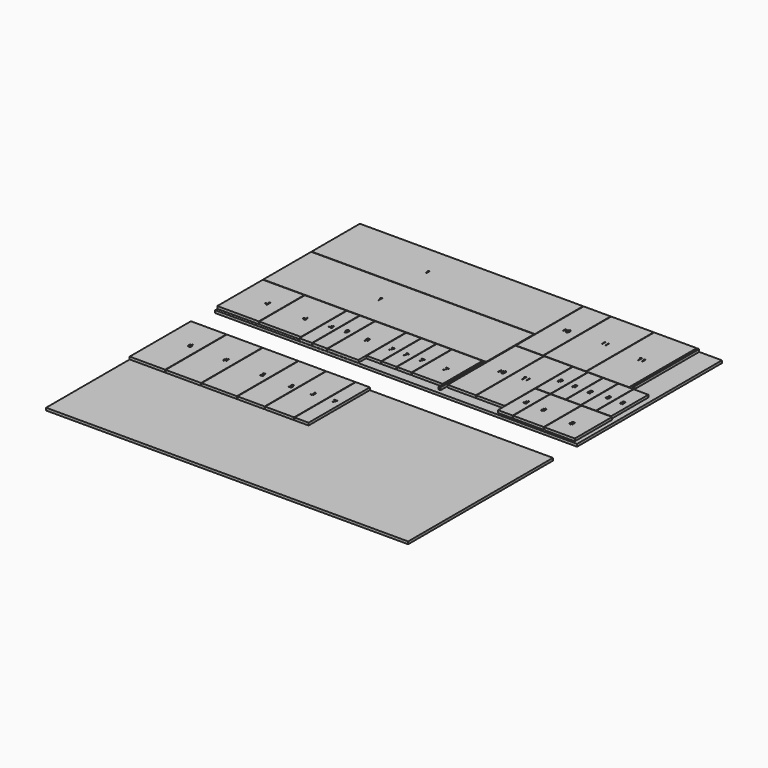
from build123d import *

# Parameters (mm, degrees)
F0_W     = 413
F0_H     = 566
F1_DEPTH = 25
F0_W_2   = 126
F0_H_2   = 591
F0_W_3   = 146
F0_W_4   = 304
F0_H_3   = 495
F0_W_5   = 20
F0_H_4   = 552
F0_W_6   = 280
F0_H_5   = 843
F0_W_7   = 2216
F0_H_6   = 596
F0_H_7   = 463
F0_W_8   = 269
F0_H_8   = 841
F0_W_9   = 422.5
F0_W_10  = 2220
F0_H_9   = 600
F0_H_10  = 802
F0_W_11  = 352.5
F0_H_11  = 761
F0_W_12  = 351
F0_W_13  = 271
F0_W_14  = 288
F0_W_15  = 139
F2_DEPTH = 25


with BuildPart() as f1:
    # F0 (on Top) → F1 (new body)
    with BuildSketch(Plane.XY):
        with Locations((-3393.5, 311)):
            Rectangle(F0_W, F0_H)
        Polygon((-3304.6911327013, 297.8236588856), (-3304.6911327013, 293.0724246738), (-3311.5159987938, 293.0724246738), (-3311.5159987938, 282.5029417872), (-3316.5188873601, 282.5029417872), (-3316.5188873601, 293.0724246738), (-3338.8859263828, 293.0724246738), (-3338.8859263828, 297.6324015763), (-3317.0523945915, 328.7469459594), (-3311.5159987938, 328.7469459594), (-3311.5159987938, 297.8236588856), align=None, mode=Mode.SUBTRACT)
    extrude(amount=F1_DEPTH)


with BuildPart() as f1b:
    # F0 (on Top) → F1, piece 2 (new body)
    with BuildSketch(Plane.XY):
        with Locations((-2975.5, 311)):
            Rectangle(F0_W, F0_H)
        Polygon((-2918.9492506751, 280.90108067), (-2918.9492506751, 276.1498464582), (-2925.7741167676, 276.1498464582), (-2925.7741167676, 265.5803635716), (-2930.7770053339, 265.5803635716), (-2930.7770053339, 276.1498464582), (-2953.1440443566, 276.1498464582), (-2953.1440443566, 280.7098233607), (-2931.3105125653, 311.8243677438), (-2925.7741167676, 311.8243677438), (-2925.7741167676, 280.90108067), align=None, mode=Mode.SUBTRACT)
    extrude(amount=F1_DEPTH)


with BuildPart() as f1c:
    # F0 (on Top) → F1, piece 3 (new body)
    with BuildSketch(Plane.XY):
        with Locations((-2701, 298.5)):
            Rectangle(F0_W_2, F0_H_2)
        Polygon((-2673.4564496049, 300.8207368871), (-2673.4564496049, 296.0695026753), (-2680.2813156974, 296.0695026753), (-2680.2813156974, 285.5000197887), (-2685.2842042637, 285.5000197887), (-2685.2842042637, 296.0695026753), (-2707.6512432864, 296.0695026753), (-2707.6512432864, 300.6294795778), (-2685.8177114951, 331.7440239609), (-2680.2813156974, 331.7440239609), (-2680.2813156974, 300.8207368871), align=None, mode=Mode.SUBTRACT)
    extrude(amount=F1_DEPTH)


with BuildPart() as f1d:
    # F0 (on Top) → F1, piece 4 (new body)
    with BuildSketch(Plane.XY):
        with Locations((-2560, 298.5)):
            Rectangle(F0_W_3, F0_H_2)
        with BuildLine():
            add(Edge.make_bspline(
                [(-2534.4639109939, 338.5323141831), (-2532.5765033356, 333.9270394968), (-2532.5765033356, 327.6658791583)],
                knots=[0, 0, 0, 1, 1, 1], degree=2))
            add(Edge.make_bspline(
                [(-2532.5765033356, 327.6658791583), (-2532.5765033356, 300.6684000138), (-2553.4638147542, 300.6684000138)],
                knots=[0, 0, 0, 1, 1, 1], degree=2))
            add(Edge.make_bspline(
                [(-2553.4638147542, 300.6684000138), (-2557.1178359807, 300.6684000138), (-2559.2518649064, 301.302568987)],
                knots=[0, 0, 0, 1, 1, 1], degree=2))
            Line((-2559.2518649064, 301.302568987), (-2559.2518649064, 305.8021488444))
            add(Edge.make_bspline(
                [(-2559.2518649064, 305.8021488444), (-2556.735321362, 304.986788736), (-2553.5342779735, 304.986788736)],
                knots=[0, 0, 0, 1, 1, 1], degree=2))
            add(Edge.make_bspline(
                [(-2553.5342779735, 304.986788736), (-2545.9846473402, 304.986788736), (-2542.1293026302, 309.6574935545)],
                knots=[0, 0, 0, 1, 1, 1], degree=2))
            add(Edge.make_bspline(
                [(-2542.1293026302, 309.6574935545), (-2538.2739579202, 314.3281983729), (-2537.9317079981, 323.9816594093)],
                knots=[0, 0, 0, 1, 1, 1], degree=2))
            Line((-2537.9317079981, 323.9816594093), (-2538.3041564427, 323.9816594093))
            add(Edge.make_bspline(
                [(-2538.3041564427, 323.9816594093), (-2540.0355384012, 321.3745202973), (-2542.8993649548, 320.0055206091)],
                knots=[0, 0, 0, 1, 1, 1], degree=2))
            add(Edge.make_bspline(
                [(-2542.8993649548, 320.0055206091), (-2545.7631915083, 318.6365209209), (-2549.3467495156, 318.6365209209)],
                knots=[0, 0, 0, 1, 1, 1], degree=2))
            add(Edge.make_bspline(
                [(-2549.3467495156, 318.6365209209), (-2555.4468510672, 318.6365209209), (-2559.0354421616, 322.2855090603)],
                knots=[0, 0, 0, 1, 1, 1], degree=2))
            add(Edge.make_bspline(
                [(-2559.0354421616, 322.2855090603), (-2562.6240332559, 325.9344971997), (-2562.6240332559, 332.4775104152)],
                knots=[0, 0, 0, 1, 1, 1], degree=2))
            add(Edge.make_bspline(
                [(-2562.6240332559, 332.4775104152), (-2562.6240332559, 339.6446264297), (-2558.6126628461, 343.796923278)],
                knots=[0, 0, 0, 1, 1, 1], degree=2))
            add(Edge.make_bspline(
                [(-2558.6126628461, 343.796923278), (-2554.6012924363, 347.9492201263), (-2548.0582792208, 347.9492201263)],
                knots=[0, 0, 0, 1, 1, 1], degree=2))
            add(Edge.make_bspline(
                [(-2548.0582792208, 347.9492201263), (-2543.3674420541, 347.9492201263), (-2539.8593803531, 345.5434044978)],
                knots=[0, 0, 0, 1, 1, 1], degree=2))
            add(Edge.make_bspline(
                [(-2539.8593803531, 345.5434044978), (-2536.3513186522, 343.1375888694), (-2534.4639109939, 338.5323141831)],
                knots=[0, 0, 0, 1, 1, 1], degree=2))
        make_face(mode=Mode.SUBTRACT)
    extrude(amount=F1_DEPTH)


with BuildPart() as f1e:
    # F0 (on Top) → F1, piece 5 (new body)
    with BuildSketch(Plane.XY):
        with Locations((-2330, 298.5)):
            Rectangle(F0_W_4, F0_H_2)
        with BuildLine():
            add(Edge.make_bspline(
                [(-2321.4638816684, 324.6067171114), (-2319.5764740101, 320.0014424252), (-2319.5764740101, 313.7402820867)],
                knots=[0, 0, 0, 1, 1, 1], degree=2))
            add(Edge.make_bspline(
                [(-2319.5764740101, 313.7402820867), (-2319.5764740101, 286.7428029422), (-2340.4637854288, 286.7428029422)],
                knots=[0, 0, 0, 1, 1, 1], degree=2))
            add(Edge.make_bspline(
                [(-2340.4637854288, 286.7428029422), (-2344.1178066553, 286.7428029422), (-2346.2518355809, 287.3769719154)],
                knots=[0, 0, 0, 1, 1, 1], degree=2))
            Line((-2346.2518355809, 287.3769719154), (-2346.2518355809, 291.8765517728))
            add(Edge.make_bspline(
                [(-2346.2518355809, 291.8765517728), (-2343.7352920365, 291.0611916644), (-2340.534248648, 291.0611916644)],
                knots=[0, 0, 0, 1, 1, 1], degree=2))
            add(Edge.make_bspline(
                [(-2340.534248648, 291.0611916644), (-2332.9846180148, 291.0611916644), (-2329.1292733047, 295.7318964828)],
                knots=[0, 0, 0, 1, 1, 1], degree=2))
            add(Edge.make_bspline(
                [(-2329.1292733047, 295.7318964828), (-2325.2739285947, 300.4026013013), (-2324.9316786726, 310.0560623376)],
                knots=[0, 0, 0, 1, 1, 1], degree=2))
            Line((-2324.9316786726, 310.0560623376), (-2325.3041271172, 310.0560623376))
            add(Edge.make_bspline(
                [(-2325.3041271172, 310.0560623376), (-2327.0355090758, 307.4489232256), (-2329.8993356293, 306.0799235375)],
                knots=[0, 0, 0, 1, 1, 1], degree=2))
            add(Edge.make_bspline(
                [(-2329.8993356293, 306.0799235375), (-2332.7631621829, 304.7109238493), (-2336.3467201901, 304.7109238493)],
                knots=[0, 0, 0, 1, 1, 1], degree=2))
            add(Edge.make_bspline(
                [(-2336.3467201901, 304.7109238493), (-2342.4468217418, 304.7109238493), (-2346.0354128361, 308.3599119887)],
                knots=[0, 0, 0, 1, 1, 1], degree=2))
            add(Edge.make_bspline(
                [(-2346.0354128361, 308.3599119887), (-2349.6240039304, 312.0089001281), (-2349.6240039304, 318.5519133436)],
                knots=[0, 0, 0, 1, 1, 1], degree=2))
            add(Edge.make_bspline(
                [(-2349.6240039304, 318.5519133436), (-2349.6240039304, 325.7190293581), (-2345.6126335206, 329.8713262064)],
                knots=[0, 0, 0, 1, 1, 1], degree=2))
            add(Edge.make_bspline(
                [(-2345.6126335206, 329.8713262064), (-2341.6012631108, 334.0236230546), (-2335.0582498954, 334.0236230546)],
                knots=[0, 0, 0, 1, 1, 1], degree=2))
            add(Edge.make_bspline(
                [(-2335.0582498954, 334.0236230546), (-2330.3674127286, 334.0236230546), (-2326.8593510277, 331.6178074262)],
                knots=[0, 0, 0, 1, 1, 1], degree=2))
            add(Edge.make_bspline(
                [(-2326.8593510277, 331.6178074262), (-2323.3512893267, 329.2119917977), (-2321.4638816684, 324.6067171114)],
                knots=[0, 0, 0, 1, 1, 1], degree=2))
        make_face(mode=Mode.SUBTRACT)
    extrude(amount=F1_DEPTH)


with BuildPart() as f1f:
    # F0 (on Top) → F1, piece 6 (new body)
    with BuildSketch(Plane.XY):
        with Locations((-2100, 346.5)):
            Rectangle(F0_W_3, F0_H_3)
        Polygon((-2094.4568176961, 286.8930995464), (-2100.2448678482, 286.8930995464), (-2081.1896001299, 328.0738181072), (-2106.2543738323, 328.0738181072), (-2106.2543738323, 332.8854493642), (-2075.6532043322, 332.8854493642), (-2075.6532043322, 328.6979209063), align=None, mode=Mode.SUBTRACT)
    extrude(amount=F1_DEPTH)


with BuildPart() as f1g:
    # F0 (on Top) → F1, piece 7 (new body)
    with BuildSketch(Plane.XY):
        with Locations((-1949, 346.5)):
            Rectangle(F0_W_3, F0_H_3)
        Polygon((-1950.243379662, 283.5497260094), (-1956.0314298142, 283.5497260094), (-1936.9761620959, 324.7304445702), (-1962.0409357982, 324.7304445702), (-1962.0409357982, 329.5420758271), (-1931.4397662982, 329.5420758271), (-1931.4397662982, 325.3545473692), align=None, mode=Mode.SUBTRACT)
    extrude(amount=F1_DEPTH)


with BuildPart() as f1h:
    # F0 (on Top) → F1, piece 8 (new body)
    with BuildSketch(Plane.XY):
        with Locations((-1798, 346.5)):
            Rectangle(F0_W_3, F0_H_3)
        Polygon((-1796.3338976002, 284.4989970326), (-1802.1219477523, 284.4989970326), (-1783.066680034, 325.6797155934), (-1808.1314537364, 325.6797155934), (-1808.1314537364, 330.4913468504), (-1777.5302842363, 330.4913468504), (-1777.5302842363, 326.3038183925), align=None, mode=Mode.SUBTRACT)
    extrude(amount=F1_DEPTH)


with BuildPart() as f1i:
    # F0 (on Top) → F1, piece 9 (new body)
    with BuildSketch(Plane.XY):
        with Locations((-1568, 346.5)):
            Rectangle(F0_W_4, F0_H_3)
        Polygon((-1556.3339253163, 284.4989970326), (-1562.1219754685, 284.4989970326), (-1543.0667077502, 325.6797155934), (-1568.1314814525, 325.6797155934), (-1568.1314814525, 330.4913468504), (-1537.5303119524, 330.4913468504), (-1537.5303119524, 326.3038183925), align=None, mode=Mode.SUBTRACT)
    extrude(amount=F1_DEPTH)


with BuildPart() as f1j:
    # F0 (on Top) → F1, piece 10 (new body)
    with BuildSketch(Plane.XY):
        with Locations((-1401, 318)):
            Rectangle(F0_W_5, F0_H_4)
    extrude(amount=F1_DEPTH)


with BuildPart() as f1k:
    # F0 (on Top) → F1, piece 11 (new body)
    with BuildSketch(Plane.XY):
        with Locations((-1235, 532.5)):
            Rectangle(F0_W_6, F0_H_5)
        with BuildLine():
            Line((-1201.2402883136, 570.3238598847), (-1201.2402883136, 524.331510067))
            Line((-1201.2402883136, 524.331510067), (-1206.3337724475, 524.331510067))
            Line((-1206.3337724475, 524.331510067), (-1206.3337724475, 557.1069731894))
            add(Edge.make_bspline(
                [(-1206.3337724475, 557.1069731894), (-1206.3337724475, 561.2039060798), (-1206.082118093, 564.8478611321)],
                knots=[0, 0, 0, 1, 1, 1], degree=2))
            add(Edge.make_bspline(
                [(-1206.082118093, 564.8478611321), (-1206.7364194146, 564.1834936363), (-1207.5568126101, 563.4637621826)],
                knots=[0, 0, 0, 1, 1, 1], degree=2))
            add(Edge.make_bspline(
                [(-1207.5568126101, 563.4637621826), (-1208.3772058055, 562.7440307289), (-1215.0410131112, 557.3284290214)],
                knots=[0, 0, 0, 1, 1, 1], degree=2))
            Line((-1215.0410131112, 557.3284290214), (-1217.80921101, 560.9119870286))
            Line((-1217.80921101, 560.9119870286), (-1205.6392064292, 570.3238598847))
            Line((-1205.6392064292, 570.3238598847), (-1201.2402883136, 570.3238598847))
        make_face(mode=Mode.SUBTRACT)
        with BuildLine():
            add(Edge.make_bspline(
                [(-1157.1504454154, 564.9736883093), (-1153.2649021829, 558.8987521931), (-1153.2649021829, 547.393115108)],
                knots=[0, 0, 0, 1, 1, 1], degree=2))
            add(Edge.make_bspline(
                [(-1153.2649021829, 547.393115108), (-1153.2649021829, 535.4646987075), (-1157.0246182382, 529.5810199006)],
                knots=[0, 0, 0, 1, 1, 1], degree=2))
            add(Edge.make_bspline(
                [(-1157.0246182382, 529.5810199006), (-1160.7843342936, 523.6973410938), (-1168.5252222362, 523.6973410938)],
                knots=[0, 0, 0, 1, 1, 1], degree=2))
            add(Edge.make_bspline(
                [(-1168.5252222362, 523.6973410938), (-1175.9439926051, 523.6973410938), (-1179.8144365764, 529.7219463391)],
                knots=[0, 0, 0, 1, 1, 1], degree=2))
            add(Edge.make_bspline(
                [(-1179.8144365764, 529.7219463391), (-1183.6848805477, 535.7465515845), (-1183.6848805477, 547.393115108)],
                knots=[0, 0, 0, 1, 1, 1], degree=2))
            add(Edge.make_bspline(
                [(-1183.6848805477, 547.393115108), (-1183.6848805477, 559.402060902), (-1179.9402637537, 565.2253426637)],
                knots=[0, 0, 0, 1, 1, 1], degree=2))
            add(Edge.make_bspline(
                [(-1179.9402637537, 565.2253426637), (-1176.1956469596, 571.0486244255), (-1168.5252222362, 571.0486244255)],
                knots=[0, 0, 0, 1, 1, 1], degree=2))
            add(Edge.make_bspline(
                [(-1168.5252222362, 571.0486244255), (-1161.035988648, 571.0486244255), (-1157.1504454154, 564.9736883093)],
                knots=[0, 0, 0, 1, 1, 1], degree=2))
        make_face(mode=Mode.SUBTRACT)
    extrude(amount=F1_DEPTH)


with BuildPart() as f1l:
    # F0 (on Top) → F1, piece 12 (new body)
    with BuildSketch(Plane.XY):
        with BuildLine():
            add(Edge.make_bspline(
                [(-1176.0396212598, 561.9739684043), (-1178.4001391045, 557.4290907631), (-1178.4001391045, 547.393115108)],
                knots=[0, 0, 0, 1, 1, 1], degree=2))
            add(Edge.make_bspline(
                [(-1178.4001391045, 547.393115108), (-1178.4001391045, 537.3571394529), (-1176.0396212598, 532.777030202)],
                knots=[0, 0, 0, 1, 1, 1], degree=2))
            add(Edge.make_bspline(
                [(-1176.0396212598, 532.777030202), (-1173.6791034151, 528.1969209512), (-1168.5252222362, 528.1969209512)],
                knots=[0, 0, 0, 1, 1, 1], degree=2))
            add(Edge.make_bspline(
                [(-1168.5252222362, 528.1969209512), (-1163.300877838, 528.1969209512), (-1160.9604923417, 532.8374272471)],
                knots=[0, 0, 0, 1, 1, 1], degree=2))
            add(Edge.make_bspline(
                [(-1160.9604923417, 532.8374272471), (-1158.6201068454, 537.477933543), (-1158.6201068454, 547.393115108)],
                knots=[0, 0, 0, 1, 1, 1], degree=2))
            add(Edge.make_bspline(
                [(-1158.6201068454, 547.393115108), (-1158.6201068454, 557.2982304988), (-1160.9604923417, 561.9085382722)],
                knots=[0, 0, 0, 1, 1, 1], degree=2))
            add(Edge.make_bspline(
                [(-1160.9604923417, 561.9085382722), (-1163.300877838, 566.5188460456), (-1168.5252222362, 566.5188460456)],
                knots=[0, 0, 0, 1, 1, 1], degree=2))
            add(Edge.make_bspline(
                [(-1168.5252222362, 566.5188460456), (-1173.6791034151, 566.5188460456), (-1176.0396212598, 561.9739684043)],
                knots=[0, 0, 0, 1, 1, 1], degree=2))
        make_face()
    extrude(amount=F1_DEPTH)


with BuildPart() as f1m:
    # F0 (on Top) → F1, piece 13 (new body)
    with BuildSketch(Plane.XY):
        with Locations((-950, 532.5)):
            Rectangle(F0_W_6, F0_H_5)
        with BuildLine():
            Line((-977.8160585427, 591.3100443625), (-977.8160585427, 545.3176945448))
            Line((-977.8160585427, 545.3176945448), (-982.9095426766, 545.3176945448))
            Line((-982.9095426766, 545.3176945448), (-982.9095426766, 578.0931576673))
            add(Edge.make_bspline(
                [(-982.9095426766, 578.0931576673), (-982.9095426766, 582.1900905576), (-982.6578883221, 585.8340456099)],
                knots=[0, 0, 0, 1, 1, 1], degree=2))
            add(Edge.make_bspline(
                [(-982.6578883221, 585.8340456099), (-983.3121896437, 585.1696781141), (-984.1325828392, 584.4499466604)],
                knots=[0, 0, 0, 1, 1, 1], degree=2))
            add(Edge.make_bspline(
                [(-984.1325828392, 584.4499466604), (-984.9529760346, 583.7302152067), (-991.6167833403, 578.3146134992)],
                knots=[0, 0, 0, 1, 1, 1], degree=2))
            Line((-991.6167833403, 578.3146134992), (-994.3849812391, 581.8981715064))
            Line((-994.3849812391, 581.8981715064), (-982.2149766583, 591.3100443625))
            Line((-982.2149766583, 591.3100443625), (-977.8160585427, 591.3100443625))
        make_face(mode=Mode.SUBTRACT)
        with BuildLine():
            Line((-940.9839272266, 591.3100443625), (-940.9839272266, 545.3176945448))
            Line((-940.9839272266, 545.3176945448), (-946.0774113605, 545.3176945448))
            Line((-946.0774113605, 545.3176945448), (-946.0774113605, 578.0931576673))
            add(Edge.make_bspline(
                [(-946.0774113605, 578.0931576673), (-946.0774113605, 582.1900905576), (-945.8257570061, 585.8340456099)],
                knots=[0, 0, 0, 1, 1, 1], degree=2))
            add(Edge.make_bspline(
                [(-945.8257570061, 585.8340456099), (-946.4800583276, 585.1696781141), (-947.3004515231, 584.4499466604)],
                knots=[0, 0, 0, 1, 1, 1], degree=2))
            add(Edge.make_bspline(
                [(-947.3004515231, 584.4499466604), (-948.1208447186, 583.7302152067), (-954.7846520242, 578.3146134992)],
                knots=[0, 0, 0, 1, 1, 1], degree=2))
            Line((-954.7846520242, 578.3146134992), (-957.5528499231, 581.8981715064))
            Line((-957.5528499231, 581.8981715064), (-945.3828453423, 591.3100443625))
            Line((-945.3828453423, 591.3100443625), (-940.9839272266, 591.3100443625))
        make_face(mode=Mode.SUBTRACT)
    extrude(amount=F1_DEPTH)


with BuildPart() as f1n:
    # F0 (on Top) → F1, piece 14 (new body)
    with BuildSketch(Plane.XY):
        with Locations((-2492, 897)):
            Rectangle(F0_W_7, F0_H_6)
        with BuildLine():
            Line((-2680.9747675951, 930.9925786996), (-2680.9747675951, 885.0002288818))
            Line((-2680.9747675951, 885.0002288818), (-2686.068251729, 885.0002288818))
            Line((-2686.068251729, 885.0002288818), (-2686.068251729, 917.7756920043))
            add(Edge.make_bspline(
                [(-2686.068251729, 917.7756920043), (-2686.068251729, 921.8726248946), (-2685.8165973746, 925.5165799469)],
                knots=[0, 0, 0, 1, 1, 1], degree=2))
            add(Edge.make_bspline(
                [(-2685.8165973746, 925.5165799469), (-2686.4708986961, 924.8522124512), (-2687.2912918916, 924.1324809975)],
                knots=[0, 0, 0, 1, 1, 1], degree=2))
            add(Edge.make_bspline(
                [(-2687.2912918916, 924.1324809975), (-2688.1116850871, 923.4127495438), (-2694.7754923927, 917.9971478362)],
                knots=[0, 0, 0, 1, 1, 1], degree=2))
            Line((-2694.7754923927, 917.9971478362), (-2697.5436902915, 921.5807058435))
            Line((-2697.5436902915, 921.5807058435), (-2685.3736857108, 930.9925786996))
            Line((-2685.3736857108, 930.9925786996), (-2680.9747675951, 930.9925786996))
        make_face(mode=Mode.SUBTRACT)
    extrude(amount=F1_DEPTH)


with BuildPart() as f1o:
    # F0 (on Top) → F1, piece 15 (new body)
    with BuildSketch(Plane.XY):
        with BuildLine():
            Line((-2702.4268988882, 300.8207368871), (-2685.2842042637, 300.8207368871))
            Line((-2685.2842042637, 300.8207368871), (-2685.2842042637, 316.111255463))
            add(Edge.make_bspline(
                [(-2685.2842042637, 316.111255463), (-2685.2842042637, 320.6108353204), (-2684.96208669, 326.2680252083)],
                knots=[0, 0, 0, 1, 1, 1], degree=2))
            Line((-2684.96208669, 326.2680252083), (-2685.2137410444, 326.2680252083))
            add(Edge.make_bspline(
                [(-2685.2137410444, 326.2680252083), (-2686.7236671711, 323.248172955), (-2688.0524021625, 321.265136642)],
                knots=[0, 0, 0, 1, 1, 1], degree=2))
            Line((-2688.0524021625, 321.265136642), (-2702.4268988882, 300.8207368871))
        make_face()
    extrude(amount=F1_DEPTH)


with BuildPart() as f1p:
    # F0 (on Top) → F1, piece 16 (new body)
    with BuildSketch(Plane.XY):
        with BuildLine():
            add(Edge.make_bspline(
                [(-2542.7584385163, 341.8843501842), (-2545.0686254901, 343.4899049656), (-2548.0582792208, 343.4899049656)],
                knots=[0, 0, 0, 1, 1, 1], degree=2))
            add(Edge.make_bspline(
                [(-2548.0582792208, 343.4899049656), (-2552.5578590783, 343.4899049656), (-2555.0089724905, 340.5958798895)],
                knots=[0, 0, 0, 1, 1, 1], degree=2))
            add(Edge.make_bspline(
                [(-2555.0089724905, 340.5958798895), (-2557.4600859028, 337.7018548134), (-2557.4600859028, 332.5379074603)],
                knots=[0, 0, 0, 1, 1, 1], degree=2))
            add(Edge.make_bspline(
                [(-2557.4600859028, 332.5379074603), (-2557.4600859028, 328.0081290803), (-2555.1951967128, 325.4160892296)],
                knots=[0, 0, 0, 1, 1, 1], degree=2))
            add(Edge.make_bspline(
                [(-2555.1951967128, 325.4160892296), (-2552.9303075228, 322.8240493788), (-2548.3099335753, 322.8240493788)],
                knots=[0, 0, 0, 1, 1, 1], degree=2))
            add(Edge.make_bspline(
                [(-2548.3099335753, 322.8240493788), (-2545.4410739347, 322.8240493788), (-2543.0352583062, 323.9866924964)],
                knots=[0, 0, 0, 1, 1, 1], degree=2))
            add(Edge.make_bspline(
                [(-2543.0352583062, 323.9866924964), (-2540.6294426777, 325.1493356139), (-2539.2453437283, 327.1625704494)],
                knots=[0, 0, 0, 1, 1, 1], degree=2))
            add(Edge.make_bspline(
                [(-2539.2453437283, 327.1625704494), (-2537.8612447789, 329.175805285), (-2537.8612447789, 331.3802974299)],
                knots=[0, 0, 0, 1, 1, 1], degree=2))
            add(Edge.make_bspline(
                [(-2537.8612447789, 331.3802974299), (-2537.8612447789, 334.6820025601), (-2539.1547481607, 337.4803989815)],
                knots=[0, 0, 0, 1, 1, 1], degree=2))
            add(Edge.make_bspline(
                [(-2539.1547481607, 337.4803989815), (-2540.4482515425, 340.2787954029), (-2542.7584385163, 341.8843501842)],
                knots=[0, 0, 0, 1, 1, 1], degree=2))
        make_face()
    extrude(amount=F1_DEPTH)


with BuildPart() as f1q:
    # F0 (on Top) → F1, piece 17 (new body)
    with BuildSketch(Plane.XY):
        with BuildLine():
            add(Edge.make_bspline(
                [(-2329.7584091908, 327.9587531126), (-2332.0685961646, 329.5643078939), (-2335.0582498954, 329.5643078939)],
                knots=[0, 0, 0, 1, 1, 1], degree=2))
            add(Edge.make_bspline(
                [(-2335.0582498954, 329.5643078939), (-2339.5578297528, 329.5643078939), (-2342.008943165, 326.6702828179)],
                knots=[0, 0, 0, 1, 1, 1], degree=2))
            add(Edge.make_bspline(
                [(-2342.008943165, 326.6702828179), (-2344.4600565773, 323.7762577418), (-2344.4600565773, 318.6123103886)],
                knots=[0, 0, 0, 1, 1, 1], degree=2))
            add(Edge.make_bspline(
                [(-2344.4600565773, 318.6123103886), (-2344.4600565773, 314.0825320087), (-2342.1951673873, 311.4904921579)],
                knots=[0, 0, 0, 1, 1, 1], degree=2))
            add(Edge.make_bspline(
                [(-2342.1951673873, 311.4904921579), (-2339.9302781973, 308.8984523072), (-2335.3099042498, 308.8984523072)],
                knots=[0, 0, 0, 1, 1, 1], degree=2))
            add(Edge.make_bspline(
                [(-2335.3099042498, 308.8984523072), (-2332.4410446092, 308.8984523072), (-2330.0352289807, 310.0610954247)],
                knots=[0, 0, 0, 1, 1, 1], degree=2))
            add(Edge.make_bspline(
                [(-2330.0352289807, 310.0610954247), (-2327.6294133522, 311.2237385422), (-2326.2453144028, 313.2369733778)],
                knots=[0, 0, 0, 1, 1, 1], degree=2))
            add(Edge.make_bspline(
                [(-2326.2453144028, 313.2369733778), (-2324.8612154534, 315.2502082133), (-2324.8612154534, 317.4547003582)],
                knots=[0, 0, 0, 1, 1, 1], degree=2))
            add(Edge.make_bspline(
                [(-2324.8612154534, 317.4547003582), (-2324.8612154534, 320.7564054885), (-2326.1547188352, 323.5548019099)],
                knots=[0, 0, 0, 1, 1, 1], degree=2))
            add(Edge.make_bspline(
                [(-2326.1547188352, 323.5548019099), (-2327.448222217, 326.3531983313), (-2329.7584091908, 327.9587531126)],
                knots=[0, 0, 0, 1, 1, 1], degree=2))
        make_face()
    extrude(amount=F1_DEPTH)


with BuildPart() as f1r:
    # F0 (on Top) → F1, piece 18 (new body)
    with BuildSketch(Plane.XY):
        with BuildLine():
            Line((-2947.9196999584, 280.90108067), (-2930.7770053339, 280.90108067))
            Line((-2930.7770053339, 280.90108067), (-2930.7770053339, 296.1915992459))
            add(Edge.make_bspline(
                [(-2930.7770053339, 296.1915992459), (-2930.7770053339, 300.6911791033), (-2930.4548877602, 306.3483689912)],
                knots=[0, 0, 0, 1, 1, 1], degree=2))
            Line((-2930.4548877602, 306.3483689912), (-2930.7065421146, 306.3483689912))
            add(Edge.make_bspline(
                [(-2930.7065421146, 306.3483689912), (-2932.2164682413, 303.3285167379), (-2933.5452032327, 301.3454804249)],
                knots=[0, 0, 0, 1, 1, 1], degree=2))
            Line((-2933.5452032327, 301.3454804249), (-2947.9196999584, 280.90108067))
        make_face()
    extrude(amount=F1_DEPTH)


with BuildPart() as f1s:
    # F0 (on Top) → F1, piece 19 (new body)
    with BuildSketch(Plane.XY):
        with BuildLine():
            Line((-3333.6615819846, 297.8236588856), (-3316.5188873601, 297.8236588856))
            Line((-3316.5188873601, 297.8236588856), (-3316.5188873601, 313.1141774615))
            add(Edge.make_bspline(
                [(-3316.5188873601, 313.1141774615), (-3316.5188873601, 317.6137573189), (-3316.1967697864, 323.2709472068)],
                knots=[0, 0, 0, 1, 1, 1], degree=2))
            Line((-3316.1967697864, 323.2709472068), (-3316.4484241408, 323.2709472068))
            add(Edge.make_bspline(
                [(-3316.4484241408, 323.2709472068), (-3317.9583502675, 320.2510949535), (-3319.2870852589, 318.2680586405)],
                knots=[0, 0, 0, 1, 1, 1], degree=2))
            Line((-3319.2870852589, 318.2680586405), (-3333.6615819846, 297.8236588856))
        make_face()
    extrude(amount=F1_DEPTH)


with BuildPart() as f1t:
    # F0 (on Top) → F1, piece 20 (new body)
    with BuildSketch(Plane.XY):
        with Locations((-732, 254.5)):
            Rectangle(F0_W_3, F0_H_7)
        with BuildLine():
            add(Edge.make_bspline(
                [(-726.5242360429, 286.4041561002), (-722.8299501197, 289.3736774826), (-716.6291868262, 289.3736774826)],
                knots=[0, 0, 0, 1, 1, 1], degree=2))
            add(Edge.make_bspline(
                [(-716.6291868262, 289.3736774826), (-710.3378279652, 289.3736774826), (-706.6586413033, 286.449453884)],
                knots=[0, 0, 0, 1, 1, 1], degree=2))
            add(Edge.make_bspline(
                [(-706.6586413033, 286.449453884), (-702.9794546413, 283.5252302854), (-702.9794546413, 278.3713491064)],
                knots=[0, 0, 0, 1, 1, 1], degree=2))
            add(Edge.make_bspline(
                [(-702.9794546413, 278.3713491064), (-702.9794546413, 274.9689822344), (-705.0832850445, 272.170585813)],
                knots=[0, 0, 0, 1, 1, 1], degree=2))
            add(Edge.make_bspline(
                [(-705.0832850445, 272.170585813), (-707.1871154476, 269.3721893916), (-711.8175555693, 267.0771016791)],
                knots=[0, 0, 0, 1, 1, 1], degree=2))
            add(Edge.make_bspline(
                [(-711.8175555693, 267.0771016791), (-706.2207627265, 264.3994993478), (-703.8602448819, 261.460176488)],
                knots=[0, 0, 0, 1, 1, 1], degree=2))
            add(Edge.make_bspline(
                [(-703.8602448819, 261.460176488), (-701.4997270372, 258.5208536281), (-701.4997270372, 254.6453765697)],
                knots=[0, 0, 0, 1, 1, 1], degree=2))
            add(Edge.make_bspline(
                [(-701.4997270372, 254.6453765697), (-701.4997270372, 248.9277896368), (-705.4959981857, 245.5103235035)],
                knots=[0, 0, 0, 1, 1, 1], degree=2))
            add(Edge.make_bspline(
                [(-705.4959981857, 245.5103235035), (-709.4922693343, 242.0928573702), (-716.4379295169, 242.0928573702)],
                knots=[0, 0, 0, 1, 1, 1], degree=2))
            add(Edge.make_bspline(
                [(-716.4379295169, 242.0928573702), (-723.7963028407, 242.0928573702), (-727.7623754667, 245.3190661941)],
                knots=[0, 0, 0, 1, 1, 1], degree=2))
            add(Edge.make_bspline(
                [(-727.7623754667, 245.3190661941), (-731.7284480927, 248.545275018), (-731.7284480927, 254.4641854345)],
                knots=[0, 0, 0, 1, 1, 1], degree=2))
            add(Edge.make_bspline(
                [(-731.7284480927, 254.4641854345), (-731.7284480927, 262.3560659898), (-722.1051855789, 266.7650502796)],
                knots=[0, 0, 0, 1, 1, 1], degree=2))
            add(Edge.make_bspline(
                [(-722.1051855789, 266.7650502796), (-726.4437066495, 269.2111306048), (-728.3311143078, 272.059857897)],
                knots=[0, 0, 0, 1, 1, 1], degree=2))
            add(Edge.make_bspline(
                [(-728.3311143078, 272.059857897), (-730.2185219661, 274.9085851893), (-730.2185219661, 278.4317461515)],
                knots=[0, 0, 0, 1, 1, 1], degree=2))
            add(Edge.make_bspline(
                [(-730.2185219661, 278.4317461515), (-730.2185219661, 283.4346347178), (-726.5242360429, 286.4041561002)],
                knots=[0, 0, 0, 1, 1, 1], degree=2))
        make_face(mode=Mode.SUBTRACT)
    extrude(amount=F1_DEPTH)


with BuildPart() as f1u:
    # F0 (on Top) → F1, piece 21 (new body)
    with BuildSketch(Plane.XY):
        with BuildLine():
            add(Edge.make_bspline(
                [(-724.4606703365, 260.1717061932), (-726.5645007396, 257.7356920422), (-726.5645007396, 254.3333251702)],
                knots=[0, 0, 0, 1, 1, 1], degree=2))
            add(Edge.make_bspline(
                [(-726.5645007396, 254.3333251702), (-726.5645007396, 250.5585098536), (-723.9422623663, 248.4496463633)],
                knots=[0, 0, 0, 1, 1, 1], degree=2))
            add(Edge.make_bspline(
                [(-723.9422623663, 248.4496463633), (-721.320023993, 246.3407828731), (-716.5687897812, 246.3407828731)],
                knots=[0, 0, 0, 1, 1, 1], degree=2))
            add(Edge.make_bspline(
                [(-716.5687897812, 246.3407828731), (-711.8779526144, 246.3407828731), (-709.2657804153, 248.545275018)],
                knots=[0, 0, 0, 1, 1, 1], degree=2))
            add(Edge.make_bspline(
                [(-709.2657804153, 248.545275018), (-706.6536082162, 250.7497671629), (-706.6536082162, 254.5849795246)],
                knots=[0, 0, 0, 1, 1, 1], degree=2))
            add(Edge.make_bspline(
                [(-706.6536082162, 254.5849795246), (-706.6536082162, 257.6350303005), (-709.1097547155, 260.0106474064)],
                knots=[0, 0, 0, 1, 1, 1], degree=2))
            add(Edge.make_bspline(
                [(-709.1097547155, 260.0106474064), (-711.5659012149, 262.3862645123), (-717.6660027665, 264.6209551798)],
                knots=[0, 0, 0, 1, 1, 1], degree=2))
            add(Edge.make_bspline(
                [(-717.6660027665, 264.6209551798), (-722.3568399333, 262.6077203442), (-724.4606703365, 260.1717061932)],
                knots=[0, 0, 0, 1, 1, 1], degree=2))
        make_face()
    extrude(amount=F1_DEPTH)


with BuildPart() as f1v:
    # F0 (on Top) → F1, piece 22 (new body)
    with BuildSketch(Plane.XY):
        with BuildLine():
            add(Edge.make_bspline(
                [(-710.4133242715, 283.2635097568), (-712.6933127228, 285.1358181538), (-716.6895838713, 285.1358181538)],
                knots=[0, 0, 0, 1, 1, 1], degree=2))
            add(Edge.make_bspline(
                [(-716.6895838713, 285.1358181538), (-720.6254579748, 285.1358181538), (-722.8601486422, 283.2484104955)],
                knots=[0, 0, 0, 1, 1, 1], degree=2))
            add(Edge.make_bspline(
                [(-722.8601486422, 283.2484104955), (-725.0948393097, 281.3610028372), (-725.0948393097, 278.2102903196)],
                knots=[0, 0, 0, 1, 1, 1], degree=2))
            add(Edge.make_bspline(
                [(-725.0948393097, 278.2102903196), (-725.0948393097, 275.3212983306), (-723.2376301739, 273.2426333629)],
                knots=[0, 0, 0, 1, 1, 1], degree=2))
            add(Edge.make_bspline(
                [(-723.2376301739, 273.2426333629), (-721.3804210381, 271.1639683952), (-716.3775324718, 269.0903365146)],
                knots=[0, 0, 0, 1, 1, 1], degree=2))
            add(Edge.make_bspline(
                [(-716.3775324718, 269.0903365146), (-711.8779526144, 270.9727110859), (-710.0056442173, 273.1470047082)],
                knots=[0, 0, 0, 1, 1, 1], degree=2))
            add(Edge.make_bspline(
                [(-710.0056442173, 273.1470047082), (-708.1333358203, 275.3212983306), (-708.1333358203, 278.2102903196)],
                knots=[0, 0, 0, 1, 1, 1], degree=2))
            add(Edge.make_bspline(
                [(-708.1333358203, 278.2102903196), (-708.1333358203, 281.3912013597), (-710.4133242715, 283.2635097568)],
                knots=[0, 0, 0, 1, 1, 1], degree=2))
        make_face()
    extrude(amount=F1_DEPTH)


with BuildPart() as f1w:
    # F0 (on Top) → F1, piece 23 (new body)
    with BuildSketch(Plane.XY):
        with Locations((-502, 254.5)):
            Rectangle(F0_W_4, F0_H_7)
        with BuildLine():
            add(Edge.make_bspline(
                [(-540.5241869287, 270.4041385764), (-536.8299010055, 273.3736599589), (-530.629137712, 273.3736599589)],
                knots=[0, 0, 0, 1, 1, 1], degree=2))
            add(Edge.make_bspline(
                [(-530.629137712, 273.3736599589), (-524.337778851, 273.3736599589), (-520.658592189, 270.4494363602)],
                knots=[0, 0, 0, 1, 1, 1], degree=2))
            add(Edge.make_bspline(
                [(-520.658592189, 270.4494363602), (-516.9794055271, 267.5252127616), (-516.9794055271, 262.3713315827)],
                knots=[0, 0, 0, 1, 1, 1], degree=2))
            add(Edge.make_bspline(
                [(-516.9794055271, 262.3713315827), (-516.9794055271, 258.9689647106), (-519.0832359302, 256.1705682892)],
                knots=[0, 0, 0, 1, 1, 1], degree=2))
            add(Edge.make_bspline(
                [(-519.0832359302, 256.1705682892), (-521.1870663334, 253.3721718678), (-525.8175064551, 251.0770841553)],
                knots=[0, 0, 0, 1, 1, 1], degree=2))
            add(Edge.make_bspline(
                [(-525.8175064551, 251.0770841553), (-520.2207136123, 248.3994818241), (-517.8601957677, 245.4601589642)],
                knots=[0, 0, 0, 1, 1, 1], degree=2))
            add(Edge.make_bspline(
                [(-517.8601957677, 245.4601589642), (-515.499677923, 242.5208361043), (-515.499677923, 238.6453590459)],
                knots=[0, 0, 0, 1, 1, 1], degree=2))
            add(Edge.make_bspline(
                [(-515.499677923, 238.6453590459), (-515.499677923, 232.927772113), (-519.4959490715, 229.5103059797)],
                knots=[0, 0, 0, 1, 1, 1], degree=2))
            add(Edge.make_bspline(
                [(-519.4959490715, 229.5103059797), (-523.4922202201, 226.0928398464), (-530.4378804026, 226.0928398464)],
                knots=[0, 0, 0, 1, 1, 1], degree=2))
            add(Edge.make_bspline(
                [(-530.4378804026, 226.0928398464), (-537.7962537265, 226.0928398464), (-541.7623263525, 229.3190486703)],
                knots=[0, 0, 0, 1, 1, 1], degree=2))
            add(Edge.make_bspline(
                [(-541.7623263525, 229.3190486703), (-545.7283989785, 232.5452574943), (-545.7283989785, 238.4641679107)],
                knots=[0, 0, 0, 1, 1, 1], degree=2))
            add(Edge.make_bspline(
                [(-545.7283989785, 238.4641679107), (-545.7283989785, 246.356048466), (-536.1051364647, 250.7650327558)],
                knots=[0, 0, 0, 1, 1, 1], degree=2))
            add(Edge.make_bspline(
                [(-536.1051364647, 250.7650327558), (-540.4436575352, 253.211113081), (-542.3310651935, 256.0598403733)],
                knots=[0, 0, 0, 1, 1, 1], degree=2))
            add(Edge.make_bspline(
                [(-542.3310651935, 256.0598403733), (-544.2184728519, 258.9085676656), (-544.2184728519, 262.4317286277)],
                knots=[0, 0, 0, 1, 1, 1], degree=2))
            add(Edge.make_bspline(
                [(-544.2184728519, 262.4317286277), (-544.2184728519, 267.434617194), (-540.5241869287, 270.4041385764)],
                knots=[0, 0, 0, 1, 1, 1], degree=2))
        make_face(mode=Mode.SUBTRACT)
    extrude(amount=F1_DEPTH)


with BuildPart() as f1x:
    # F0 (on Top) → F1, piece 24 (new body)
    with BuildSketch(Plane.XY):
        with BuildLine():
            add(Edge.make_bspline(
                [(-538.4606212222, 244.1716886695), (-540.5644516254, 241.7356745185), (-540.5644516254, 238.3333076464)],
                knots=[0, 0, 0, 1, 1, 1], degree=2))
            add(Edge.make_bspline(
                [(-540.5644516254, 238.3333076464), (-540.5644516254, 234.5584923298), (-537.9422132521, 232.4496288396)],
                knots=[0, 0, 0, 1, 1, 1], degree=2))
            add(Edge.make_bspline(
                [(-537.9422132521, 232.4496288396), (-535.3199748788, 230.3407653494), (-530.5687406669, 230.3407653494)],
                knots=[0, 0, 0, 1, 1, 1], degree=2))
            add(Edge.make_bspline(
                [(-530.5687406669, 230.3407653494), (-525.8779035002, 230.3407653494), (-523.2657313011, 232.5452574943)],
                knots=[0, 0, 0, 1, 1, 1], degree=2))
            add(Edge.make_bspline(
                [(-523.2657313011, 232.5452574943), (-520.653559102, 234.7497496392), (-520.653559102, 238.5849620009)],
                knots=[0, 0, 0, 1, 1, 1], degree=2))
            add(Edge.make_bspline(
                [(-520.653559102, 238.5849620009), (-520.653559102, 241.6350127767), (-523.1097056013, 244.0106298826)],
                knots=[0, 0, 0, 1, 1, 1], degree=2))
            add(Edge.make_bspline(
                [(-523.1097056013, 244.0106298826), (-525.5658521007, 246.3862469885), (-531.6659536523, 248.620937656)],
                knots=[0, 0, 0, 1, 1, 1], degree=2))
            add(Edge.make_bspline(
                [(-531.6659536523, 248.620937656), (-536.3567908191, 246.6077028205), (-538.4606212222, 244.1716886695)],
                knots=[0, 0, 0, 1, 1, 1], degree=2))
        make_face()
    extrude(amount=F1_DEPTH)


with BuildPart() as f1y:
    # F0 (on Top) → F1, piece 25 (new body)
    with BuildSketch(Plane.XY):
        with BuildLine():
            add(Edge.make_bspline(
                [(-524.4132751573, 267.263492233), (-526.6932636085, 269.1358006301), (-530.6895347571, 269.1358006301)],
                knots=[0, 0, 0, 1, 1, 1], degree=2))
            add(Edge.make_bspline(
                [(-530.6895347571, 269.1358006301), (-534.6254088605, 269.1358006301), (-536.860099528, 267.2483929717)],
                knots=[0, 0, 0, 1, 1, 1], degree=2))
            add(Edge.make_bspline(
                [(-536.860099528, 267.2483929717), (-539.0947901954, 265.3609853134), (-539.0947901954, 262.2102727958)],
                knots=[0, 0, 0, 1, 1, 1], degree=2))
            add(Edge.make_bspline(
                [(-539.0947901954, 262.2102727958), (-539.0947901954, 259.3212808068), (-537.2375810596, 257.2426158392)],
                knots=[0, 0, 0, 1, 1, 1], degree=2))
            add(Edge.make_bspline(
                [(-537.2375810596, 257.2426158392), (-535.3803719239, 255.1639508715), (-530.3774833576, 253.0903189909)],
                knots=[0, 0, 0, 1, 1, 1], degree=2))
            add(Edge.make_bspline(
                [(-530.3774833576, 253.0903189909), (-525.8779035002, 254.9726935621), (-524.0055951031, 257.1469871845)],
                knots=[0, 0, 0, 1, 1, 1], degree=2))
            add(Edge.make_bspline(
                [(-524.0055951031, 257.1469871845), (-522.1332867061, 259.3212808068), (-522.1332867061, 262.2102727958)],
                knots=[0, 0, 0, 1, 1, 1], degree=2))
            add(Edge.make_bspline(
                [(-522.1332867061, 262.2102727958), (-522.1332867061, 265.391183836), (-524.4132751573, 267.263492233)],
                knots=[0, 0, 0, 1, 1, 1], degree=2))
        make_face()
    extrude(amount=F1_DEPTH)


with BuildPart() as f1z:
    # F0 (on Top) → F1, piece 26 (new body)
    with BuildSketch(Plane.XY):
        with Locations((-193, 254.5)):
            Rectangle(F0_W_4, F0_H_7)
        with BuildLine():
            add(Edge.make_bspline(
                [(-226.6315393046, 229.8097396011), (-222.9372533814, 232.7792609835), (-216.736490088, 232.7792609835)],
                knots=[0, 0, 0, 1, 1, 1], degree=2))
            add(Edge.make_bspline(
                [(-216.736490088, 232.7792609835), (-210.445131227, 232.7792609835), (-206.765944565, 229.8550373849)],
                knots=[0, 0, 0, 1, 1, 1], degree=2))
            add(Edge.make_bspline(
                [(-206.765944565, 229.8550373849), (-203.0867579031, 226.9308137863), (-203.0867579031, 221.7769326073)],
                knots=[0, 0, 0, 1, 1, 1], degree=2))
            add(Edge.make_bspline(
                [(-203.0867579031, 221.7769326073), (-203.0867579031, 218.3745657353), (-205.1905883062, 215.5761693139)],
                knots=[0, 0, 0, 1, 1, 1], degree=2))
            add(Edge.make_bspline(
                [(-205.1905883062, 215.5761693139), (-207.2944187094, 212.7777728925), (-211.9248588311, 210.48268518)],
                knots=[0, 0, 0, 1, 1, 1], degree=2))
            add(Edge.make_bspline(
                [(-211.9248588311, 210.48268518), (-206.3280659883, 207.8050828487), (-203.9675481436, 204.8657599888)],
                knots=[0, 0, 0, 1, 1, 1], degree=2))
            add(Edge.make_bspline(
                [(-203.9675481436, 204.8657599888), (-201.607030299, 201.926437129), (-201.607030299, 198.0509600706)],
                knots=[0, 0, 0, 1, 1, 1], degree=2))
            add(Edge.make_bspline(
                [(-201.607030299, 198.0509600706), (-201.607030299, 192.3333731376), (-205.6033014475, 188.9159070043)],
                knots=[0, 0, 0, 1, 1, 1], degree=2))
            add(Edge.make_bspline(
                [(-205.6033014475, 188.9159070043), (-209.599572596, 185.498440871), (-216.5452327786, 185.498440871)],
                knots=[0, 0, 0, 1, 1, 1], degree=2))
            add(Edge.make_bspline(
                [(-216.5452327786, 185.498440871), (-223.9036061025, 185.498440871), (-227.8696787285, 188.724649695)],
                knots=[0, 0, 0, 1, 1, 1], degree=2))
            add(Edge.make_bspline(
                [(-227.8696787285, 188.724649695), (-231.8357513545, 191.9508585189), (-231.8357513545, 197.8697689354)],
                knots=[0, 0, 0, 1, 1, 1], degree=2))
            add(Edge.make_bspline(
                [(-231.8357513545, 197.8697689354), (-231.8357513545, 205.7616494906), (-222.2124888406, 210.1706337805)],
                knots=[0, 0, 0, 1, 1, 1], degree=2))
            add(Edge.make_bspline(
                [(-222.2124888406, 210.1706337805), (-226.5510099112, 212.6167141056), (-228.4384175695, 215.4654413979)],
                knots=[0, 0, 0, 1, 1, 1], degree=2))
            add(Edge.make_bspline(
                [(-228.4384175695, 215.4654413979), (-230.3258252278, 218.3141686902), (-230.3258252278, 221.8373296524)],
                knots=[0, 0, 0, 1, 1, 1], degree=2))
            add(Edge.make_bspline(
                [(-230.3258252278, 221.8373296524), (-230.3258252278, 226.8402182187), (-226.6315393046, 229.8097396011)],
                knots=[0, 0, 0, 1, 1, 1], degree=2))
        make_face(mode=Mode.SUBTRACT)
    extrude(amount=F1_DEPTH)


with BuildPart() as f1ba:
    # F0 (on Top) → F1, piece 27 (new body)
    with BuildSketch(Plane.XY):
        with BuildLine():
            add(Edge.make_bspline(
                [(-224.5679735982, 203.5772896941), (-226.6718040013, 201.1412755431), (-226.6718040013, 197.738908671)],
                knots=[0, 0, 0, 1, 1, 1], degree=2))
            add(Edge.make_bspline(
                [(-226.6718040013, 197.738908671), (-226.6718040013, 193.9640933544), (-224.0495656281, 191.8552298642)],
                knots=[0, 0, 0, 1, 1, 1], degree=2))
            add(Edge.make_bspline(
                [(-224.0495656281, 191.8552298642), (-221.4273272548, 189.746366374), (-216.6760930429, 189.746366374)],
                knots=[0, 0, 0, 1, 1, 1], degree=2))
            add(Edge.make_bspline(
                [(-216.6760930429, 189.746366374), (-211.9852558761, 189.746366374), (-209.373083677, 191.9508585189)],
                knots=[0, 0, 0, 1, 1, 1], degree=2))
            add(Edge.make_bspline(
                [(-209.373083677, 191.9508585189), (-206.7609114779, 194.1553506638), (-206.7609114779, 197.9905630255)],
                knots=[0, 0, 0, 1, 1, 1], degree=2))
            add(Edge.make_bspline(
                [(-206.7609114779, 197.9905630255), (-206.7609114779, 201.0406138013), (-209.2170579773, 203.4162309072)],
                knots=[0, 0, 0, 1, 1, 1], degree=2))
            add(Edge.make_bspline(
                [(-209.2170579773, 203.4162309072), (-211.6732044766, 205.7918480132), (-217.7733060283, 208.0265386806)],
                knots=[0, 0, 0, 1, 1, 1], degree=2))
            add(Edge.make_bspline(
                [(-217.7733060283, 208.0265386806), (-222.4641431951, 206.0133038451), (-224.5679735982, 203.5772896941)],
                knots=[0, 0, 0, 1, 1, 1], degree=2))
        make_face()
    extrude(amount=F1_DEPTH)


with BuildPart() as f1bb:
    # F0 (on Top) → F1, piece 28 (new body)
    with BuildSketch(Plane.XY):
        with BuildLine():
            add(Edge.make_bspline(
                [(-210.5206275333, 226.6690932576), (-212.8006159845, 228.5414016547), (-216.7968871331, 228.5414016547)],
                knots=[0, 0, 0, 1, 1, 1], degree=2))
            add(Edge.make_bspline(
                [(-216.7968871331, 228.5414016547), (-220.7327612365, 228.5414016547), (-222.967451904, 226.6539939964)],
                knots=[0, 0, 0, 1, 1, 1], degree=2))
            add(Edge.make_bspline(
                [(-222.967451904, 226.6539939964), (-225.2021425714, 224.7665863381), (-225.2021425714, 221.6158738205)],
                knots=[0, 0, 0, 1, 1, 1], degree=2))
            add(Edge.make_bspline(
                [(-225.2021425714, 221.6158738205), (-225.2021425714, 218.7268818315), (-223.3449334356, 216.6482168638)],
                knots=[0, 0, 0, 1, 1, 1], degree=2))
            add(Edge.make_bspline(
                [(-223.3449334356, 216.6482168638), (-221.4877242999, 214.5695518961), (-216.4848357336, 212.4959200155)],
                knots=[0, 0, 0, 1, 1, 1], degree=2))
            add(Edge.make_bspline(
                [(-216.4848357336, 212.4959200155), (-211.9852558761, 214.3782945867), (-210.1129474791, 216.5525882091)],
                knots=[0, 0, 0, 1, 1, 1], degree=2))
            add(Edge.make_bspline(
                [(-210.1129474791, 216.5525882091), (-208.2406390821, 218.7268818315), (-208.2406390821, 221.6158738205)],
                knots=[0, 0, 0, 1, 1, 1], degree=2))
            add(Edge.make_bspline(
                [(-208.2406390821, 221.6158738205), (-208.2406390821, 224.7967848606), (-210.5206275333, 226.6690932576)],
                knots=[0, 0, 0, 1, 1, 1], degree=2))
        make_face()
    extrude(amount=F1_DEPTH)


with BuildPart() as f1bc:
    # F0 (on Top) → F1, piece 29 (new body)
    with BuildSketch(Plane.XY):
        with Locations((-128, 722.5)):
            Rectangle(F0_W_3, F0_H_7)
        with BuildLine():
            add(Edge.make_bspline(
                [(-133.8226221398, 742.6432603711), (-130.1283362166, 745.6127817536), (-123.9275729232, 745.6127817536)],
                knots=[0, 0, 0, 1, 1, 1], degree=2))
            add(Edge.make_bspline(
                [(-123.9275729232, 745.6127817536), (-117.6362140622, 745.6127817536), (-113.9570274002, 742.6885581549)],
                knots=[0, 0, 0, 1, 1, 1], degree=2))
            add(Edge.make_bspline(
                [(-113.9570274002, 742.6885581549), (-110.2778407383, 739.7643345563), (-110.2778407383, 734.6104533774)],
                knots=[0, 0, 0, 1, 1, 1], degree=2))
            add(Edge.make_bspline(
                [(-110.2778407383, 734.6104533774), (-110.2778407383, 731.2080865053), (-112.3816711414, 728.4096900839)],
                knots=[0, 0, 0, 1, 1, 1], degree=2))
            add(Edge.make_bspline(
                [(-112.3816711414, 728.4096900839), (-114.4855015446, 725.6112936625), (-119.1159416663, 723.31620595)],
                knots=[0, 0, 0, 1, 1, 1], degree=2))
            add(Edge.make_bspline(
                [(-119.1159416663, 723.31620595), (-113.5191488235, 720.6386036188), (-111.1586309788, 717.6992807589)],
                knots=[0, 0, 0, 1, 1, 1], degree=2))
            add(Edge.make_bspline(
                [(-111.1586309788, 717.6992807589), (-108.7981131342, 714.759957899), (-108.7981131342, 710.8844808406)],
                knots=[0, 0, 0, 1, 1, 1], degree=2))
            add(Edge.make_bspline(
                [(-108.7981131342, 710.8844808406), (-108.7981131342, 705.1668939077), (-112.7943842827, 701.7494277744)],
                knots=[0, 0, 0, 1, 1, 1], degree=2))
            add(Edge.make_bspline(
                [(-112.7943842827, 701.7494277744), (-116.7906554312, 698.3319616411), (-123.7363156138, 698.3319616411)],
                knots=[0, 0, 0, 1, 1, 1], degree=2))
            add(Edge.make_bspline(
                [(-123.7363156138, 698.3319616411), (-131.0946889377, 698.3319616411), (-135.0607615637, 701.558170465)],
                knots=[0, 0, 0, 1, 1, 1], degree=2))
            add(Edge.make_bspline(
                [(-135.0607615637, 701.558170465), (-139.0268341897, 704.784379289), (-139.0268341897, 710.7032897054)],
                knots=[0, 0, 0, 1, 1, 1], degree=2))
            add(Edge.make_bspline(
                [(-139.0268341897, 710.7032897054), (-139.0268341897, 718.5951702607), (-129.4035716758, 723.0041545505)],
                knots=[0, 0, 0, 1, 1, 1], degree=2))
            add(Edge.make_bspline(
                [(-129.4035716758, 723.0041545505), (-133.7420927464, 725.4502348757), (-135.6295004047, 728.298962168)],
                knots=[0, 0, 0, 1, 1, 1], degree=2))
            add(Edge.make_bspline(
                [(-135.6295004047, 728.298962168), (-137.516908063, 731.1476894603), (-137.516908063, 734.6708504224)],
                knots=[0, 0, 0, 1, 1, 1], degree=2))
            add(Edge.make_bspline(
                [(-137.516908063, 734.6708504224), (-137.516908063, 739.6737389887), (-133.8226221398, 742.6432603711)],
                knots=[0, 0, 0, 1, 1, 1], degree=2))
        make_face(mode=Mode.SUBTRACT)
    extrude(amount=F1_DEPTH)


with BuildPart() as f1bd:
    # F0 (on Top) → F1, piece 30 (new body)
    with BuildSketch(Plane.XY):
        with Locations((-279, 722.5)):
            Rectangle(F0_W_3, F0_H_7)
        with BuildLine():
            add(Edge.make_bspline(
                [(-278.0360601739, 745.9866339082), (-274.3417742507, 748.9561552906), (-268.1410109573, 748.9561552906)],
                knots=[0, 0, 0, 1, 1, 1], degree=2))
            add(Edge.make_bspline(
                [(-268.1410109573, 748.9561552906), (-261.8496520962, 748.9561552906), (-258.1704654343, 746.031931692)],
                knots=[0, 0, 0, 1, 1, 1], degree=2))
            add(Edge.make_bspline(
                [(-258.1704654343, 746.031931692), (-254.4912787723, 743.1077080934), (-254.4912787723, 737.9538269144)],
                knots=[0, 0, 0, 1, 1, 1], degree=2))
            add(Edge.make_bspline(
                [(-254.4912787723, 737.9538269144), (-254.4912787723, 734.5514600424), (-256.5951091755, 731.753063621)],
                knots=[0, 0, 0, 1, 1, 1], degree=2))
            add(Edge.make_bspline(
                [(-256.5951091755, 731.753063621), (-258.6989395786, 728.9546671996), (-263.3293797003, 726.6595794871)],
                knots=[0, 0, 0, 1, 1, 1], degree=2))
            add(Edge.make_bspline(
                [(-263.3293797003, 726.6595794871), (-257.7325868576, 723.9819771558), (-255.3720690129, 721.042654296)],
                knots=[0, 0, 0, 1, 1, 1], degree=2))
            add(Edge.make_bspline(
                [(-255.3720690129, 721.042654296), (-253.0115511682, 718.1033314361), (-253.0115511682, 714.2278543777)],
                knots=[0, 0, 0, 1, 1, 1], degree=2))
            add(Edge.make_bspline(
                [(-253.0115511682, 714.2278543777), (-253.0115511682, 708.5102674448), (-257.0078223168, 705.0928013115)],
                knots=[0, 0, 0, 1, 1, 1], degree=2))
            add(Edge.make_bspline(
                [(-257.0078223168, 705.0928013115), (-261.0040934653, 701.6753351782), (-267.9497536479, 701.6753351782)],
                knots=[0, 0, 0, 1, 1, 1], degree=2))
            add(Edge.make_bspline(
                [(-267.9497536479, 701.6753351782), (-275.3081269717, 701.6753351782), (-279.2741995977, 704.9015440021)],
                knots=[0, 0, 0, 1, 1, 1], degree=2))
            add(Edge.make_bspline(
                [(-279.2741995977, 704.9015440021), (-283.2402722237, 708.127752826), (-283.2402722237, 714.0466632425)],
                knots=[0, 0, 0, 1, 1, 1], degree=2))
            add(Edge.make_bspline(
                [(-283.2402722237, 714.0466632425), (-283.2402722237, 721.9385437978), (-273.6170097099, 726.3475280876)],
                knots=[0, 0, 0, 1, 1, 1], degree=2))
            add(Edge.make_bspline(
                [(-273.6170097099, 726.3475280876), (-277.9555307805, 728.7936084128), (-279.8429384388, 731.642335705)],
                knots=[0, 0, 0, 1, 1, 1], degree=2))
            add(Edge.make_bspline(
                [(-279.8429384388, 731.642335705), (-281.7303460971, 734.4910629973), (-281.7303460971, 738.0142239595)],
                knots=[0, 0, 0, 1, 1, 1], degree=2))
            add(Edge.make_bspline(
                [(-281.7303460971, 738.0142239595), (-281.7303460971, 743.0171125258), (-278.0360601739, 745.9866339082)],
                knots=[0, 0, 0, 1, 1, 1], degree=2))
        make_face(mode=Mode.SUBTRACT)
    extrude(amount=F1_DEPTH)


with BuildPart() as f1be:
    # F0 (on Top) → F1, piece 31 (new body)
    with BuildSketch(Plane.XY):
        with Locations((-430, 722.5)):
            Rectangle(F0_W_3, F0_H_7)
        with BuildLine():
            add(Edge.make_bspline(
                [(-445.5328829483, 728.3344724888), (-441.8385970251, 731.3039938712), (-435.6378337317, 731.3039938712)],
                knots=[0, 0, 0, 1, 1, 1], degree=2))
            add(Edge.make_bspline(
                [(-435.6378337317, 731.3039938712), (-429.3464748706, 731.3039938712), (-425.6672882087, 728.3797702726)],
                knots=[0, 0, 0, 1, 1, 1], degree=2))
            add(Edge.make_bspline(
                [(-425.6672882087, 728.3797702726), (-421.9881015468, 725.455546674), (-421.9881015468, 720.301665495)],
                knots=[0, 0, 0, 1, 1, 1], degree=2))
            add(Edge.make_bspline(
                [(-421.9881015468, 720.301665495), (-421.9881015468, 716.899298623), (-424.0919319499, 714.1009022016)],
                knots=[0, 0, 0, 1, 1, 1], degree=2))
            add(Edge.make_bspline(
                [(-424.0919319499, 714.1009022016), (-426.195762353, 711.3025057802), (-430.8262024747, 709.0074180677)],
                knots=[0, 0, 0, 1, 1, 1], degree=2))
            add(Edge.make_bspline(
                [(-430.8262024747, 709.0074180677), (-425.229409632, 706.3298157365), (-422.8688917873, 703.3904928766)],
                knots=[0, 0, 0, 1, 1, 1], degree=2))
            add(Edge.make_bspline(
                [(-422.8688917873, 703.3904928766), (-420.5083739426, 700.4511700167), (-420.5083739426, 696.5756929583)],
                knots=[0, 0, 0, 1, 1, 1], degree=2))
            add(Edge.make_bspline(
                [(-420.5083739426, 696.5756929583), (-420.5083739426, 690.8581060254), (-424.5046450912, 687.4406398921)],
                knots=[0, 0, 0, 1, 1, 1], degree=2))
            add(Edge.make_bspline(
                [(-424.5046450912, 687.4406398921), (-428.5009162397, 684.0231737588), (-435.4465764223, 684.0231737588)],
                knots=[0, 0, 0, 1, 1, 1], degree=2))
            add(Edge.make_bspline(
                [(-435.4465764223, 684.0231737588), (-442.8049497462, 684.0231737588), (-446.7710223722, 687.2493825827)],
                knots=[0, 0, 0, 1, 1, 1], degree=2))
            add(Edge.make_bspline(
                [(-446.7710223722, 687.2493825827), (-450.7370949982, 690.4755914066), (-450.7370949982, 696.3945018231)],
                knots=[0, 0, 0, 1, 1, 1], degree=2))
            add(Edge.make_bspline(
                [(-450.7370949982, 696.3945018231), (-450.7370949982, 704.2863823784), (-441.1138324843, 708.6953666682)],
                knots=[0, 0, 0, 1, 1, 1], degree=2))
            add(Edge.make_bspline(
                [(-441.1138324843, 708.6953666682), (-445.4523535549, 711.1414469934), (-447.3397612132, 713.9901742857)],
                knots=[0, 0, 0, 1, 1, 1], degree=2))
            add(Edge.make_bspline(
                [(-447.3397612132, 713.9901742857), (-449.2271688715, 716.8389015779), (-449.2271688715, 720.3620625401)],
                knots=[0, 0, 0, 1, 1, 1], degree=2))
            add(Edge.make_bspline(
                [(-449.2271688715, 720.3620625401), (-449.2271688715, 725.3649511064), (-445.5328829483, 728.3344724888)],
                knots=[0, 0, 0, 1, 1, 1], degree=2))
        make_face(mode=Mode.SUBTRACT)
    extrude(amount=F1_DEPTH)


with BuildPart() as f1bf:
    # F0 (on Top) → F1, piece 32 (new body)
    with BuildSketch(Plane.XY):
        with Locations((-581, 722.5)):
            Rectangle(F0_W_3, F0_H_7)
        with BuildLine():
            add(Edge.make_bspline(
                [(-599.4423650102, 727.3852014655), (-595.748079087, 730.354722848), (-589.5473157935, 730.354722848)],
                knots=[0, 0, 0, 1, 1, 1], degree=2))
            add(Edge.make_bspline(
                [(-589.5473157935, 730.354722848), (-583.2559569325, 730.354722848), (-579.5767702706, 727.4304992493)],
                knots=[0, 0, 0, 1, 1, 1], degree=2))
            add(Edge.make_bspline(
                [(-579.5767702706, 727.4304992493), (-575.8975836086, 724.5062756507), (-575.8975836086, 719.3523944718)],
                knots=[0, 0, 0, 1, 1, 1], degree=2))
            add(Edge.make_bspline(
                [(-575.8975836086, 719.3523944718), (-575.8975836086, 715.9500275997), (-578.0014140117, 713.1516311783)],
                knots=[0, 0, 0, 1, 1, 1], degree=2))
            add(Edge.make_bspline(
                [(-578.0014140117, 713.1516311783), (-580.1052444149, 710.3532347569), (-584.7356845366, 708.0581470444)],
                knots=[0, 0, 0, 1, 1, 1], degree=2))
            add(Edge.make_bspline(
                [(-584.7356845366, 708.0581470444), (-579.1388916938, 705.3805447132), (-576.7783738492, 702.4412218533)],
                knots=[0, 0, 0, 1, 1, 1], degree=2))
            add(Edge.make_bspline(
                [(-576.7783738492, 702.4412218533), (-574.4178560045, 699.5018989934), (-574.4178560045, 695.626421935)],
                knots=[0, 0, 0, 1, 1, 1], degree=2))
            add(Edge.make_bspline(
                [(-574.4178560045, 695.626421935), (-574.4178560045, 689.9088350021), (-578.414127153, 686.4913688688)],
                knots=[0, 0, 0, 1, 1, 1], degree=2))
            add(Edge.make_bspline(
                [(-578.414127153, 686.4913688688), (-582.4103983016, 683.0739027355), (-589.3560584842, 683.0739027355)],
                knots=[0, 0, 0, 1, 1, 1], degree=2))
            add(Edge.make_bspline(
                [(-589.3560584842, 683.0739027355), (-596.714431808, 683.0739027355), (-600.680504434, 686.3001115594)],
                knots=[0, 0, 0, 1, 1, 1], degree=2))
            add(Edge.make_bspline(
                [(-600.680504434, 686.3001115594), (-604.64657706, 689.5263203834), (-604.64657706, 695.4452307998)],
                knots=[0, 0, 0, 1, 1, 1], degree=2))
            add(Edge.make_bspline(
                [(-604.64657706, 695.4452307998), (-604.64657706, 703.3371113551), (-595.0233145462, 707.7460956449)],
                knots=[0, 0, 0, 1, 1, 1], degree=2))
            add(Edge.make_bspline(
                [(-595.0233145462, 707.7460956449), (-599.3618356167, 710.1921759701), (-601.2492432751, 713.0409032624)],
                knots=[0, 0, 0, 1, 1, 1], degree=2))
            add(Edge.make_bspline(
                [(-601.2492432751, 713.0409032624), (-603.1366509334, 715.8896305547), (-603.1366509334, 719.4127915168)],
                knots=[0, 0, 0, 1, 1, 1], degree=2))
            add(Edge.make_bspline(
                [(-603.1366509334, 719.4127915168), (-603.1366509334, 724.4156800831), (-599.4423650102, 727.3852014655)],
                knots=[0, 0, 0, 1, 1, 1], degree=2))
        make_face(mode=Mode.SUBTRACT)
    extrude(amount=F1_DEPTH)


with BuildPart() as f1bg:
    # F0 (on Top) → F1, piece 33 (new body)
    with BuildSketch(Plane.XY):
        with Locations((-732, 722.5)):
            Rectangle(F0_W_3, F0_H_7)
        with BuildLine():
            add(Edge.make_bspline(
                [(-743.6558030442, 730.7285750026), (-739.961517121, 733.698096385), (-733.7607538276, 733.698096385)],
                knots=[0, 0, 0, 1, 1, 1], degree=2))
            add(Edge.make_bspline(
                [(-733.7607538276, 733.698096385), (-727.4693949665, 733.698096385), (-723.7902083046, 730.7738727864)],
                knots=[0, 0, 0, 1, 1, 1], degree=2))
            add(Edge.make_bspline(
                [(-723.7902083046, 730.7738727864), (-720.1110216427, 727.8496491878), (-720.1110216427, 722.6957680088)],
                knots=[0, 0, 0, 1, 1, 1], degree=2))
            add(Edge.make_bspline(
                [(-720.1110216427, 722.6957680088), (-720.1110216427, 719.2934011368), (-722.2148520458, 716.4950047154)],
                knots=[0, 0, 0, 1, 1, 1], degree=2))
            add(Edge.make_bspline(
                [(-722.2148520458, 716.4950047154), (-724.3186824489, 713.696608294), (-728.9491225707, 711.4015205815)],
                knots=[0, 0, 0, 1, 1, 1], degree=2))
            add(Edge.make_bspline(
                [(-728.9491225707, 711.4015205815), (-723.3523297279, 708.7239182502), (-720.9918118832, 705.7845953904)],
                knots=[0, 0, 0, 1, 1, 1], degree=2))
            add(Edge.make_bspline(
                [(-720.9918118832, 705.7845953904), (-718.6312940386, 702.8452725305), (-718.6312940386, 698.9697954721)],
                knots=[0, 0, 0, 1, 1, 1], degree=2))
            add(Edge.make_bspline(
                [(-718.6312940386, 698.9697954721), (-718.6312940386, 693.2522085392), (-722.6275651871, 689.8347424059)],
                knots=[0, 0, 0, 1, 1, 1], degree=2))
            add(Edge.make_bspline(
                [(-722.6275651871, 689.8347424059), (-726.6238363356, 686.4172762726), (-733.5694965182, 686.4172762726)],
                knots=[0, 0, 0, 1, 1, 1], degree=2))
            add(Edge.make_bspline(
                [(-733.5694965182, 686.4172762726), (-740.9278698421, 686.4172762726), (-744.8939424681, 689.6434850965)],
                knots=[0, 0, 0, 1, 1, 1], degree=2))
            add(Edge.make_bspline(
                [(-744.8939424681, 689.6434850965), (-748.8600150941, 692.8696939204), (-748.8600150941, 698.7886043369)],
                knots=[0, 0, 0, 1, 1, 1], degree=2))
            add(Edge.make_bspline(
                [(-748.8600150941, 698.7886043369), (-748.8600150941, 706.6804848922), (-739.2367525802, 711.089469182)],
                knots=[0, 0, 0, 1, 1, 1], degree=2))
            add(Edge.make_bspline(
                [(-739.2367525802, 711.089469182), (-743.5752736508, 713.5355495072), (-745.4626813091, 716.3842767994)],
                knots=[0, 0, 0, 1, 1, 1], degree=2))
            add(Edge.make_bspline(
                [(-745.4626813091, 716.3842767994), (-747.3500889674, 719.2330040917), (-747.3500889674, 722.7561650539)],
                knots=[0, 0, 0, 1, 1, 1], degree=2))
            add(Edge.make_bspline(
                [(-747.3500889674, 722.7561650539), (-747.3500889674, 727.7590536202), (-743.6558030442, 730.7285750026)],
                knots=[0, 0, 0, 1, 1, 1], degree=2))
        make_face(mode=Mode.SUBTRACT)
    extrude(amount=F1_DEPTH)


with BuildPart() as f1bh:
    # F0 (on Top) → F1, piece 34 (new body)
    with BuildSketch(Plane.XY):
        with BuildLine():
            add(Edge.make_bspline(
                [(-727.5448912729, 727.5879286592), (-729.8248797241, 729.4602370562), (-733.8211508726, 729.4602370562)],
                knots=[0, 0, 0, 1, 1, 1], degree=2))
            add(Edge.make_bspline(
                [(-733.8211508726, 729.4602370562), (-737.7570249761, 729.4602370562), (-739.9917156436, 727.5728293979)],
                knots=[0, 0, 0, 1, 1, 1], degree=2))
            add(Edge.make_bspline(
                [(-739.9917156436, 727.5728293979), (-742.226406311, 725.6854217396), (-742.226406311, 722.534709222)],
                knots=[0, 0, 0, 1, 1, 1], degree=2))
            add(Edge.make_bspline(
                [(-742.226406311, 722.534709222), (-742.226406311, 719.645717233), (-740.3691971752, 717.5670522653)],
                knots=[0, 0, 0, 1, 1, 1], degree=2))
            add(Edge.make_bspline(
                [(-740.3691971752, 717.5670522653), (-738.5119880394, 715.4883872976), (-733.5090994731, 713.414755417)],
                knots=[0, 0, 0, 1, 1, 1], degree=2))
            add(Edge.make_bspline(
                [(-733.5090994731, 713.414755417), (-729.0095196157, 715.2971299883), (-727.1372112187, 717.4714236106)],
                knots=[0, 0, 0, 1, 1, 1], degree=2))
            add(Edge.make_bspline(
                [(-727.1372112187, 717.4714236106), (-725.2649028216, 719.645717233), (-725.2649028216, 722.534709222)],
                knots=[0, 0, 0, 1, 1, 1], degree=2))
            add(Edge.make_bspline(
                [(-725.2649028216, 722.534709222), (-725.2649028216, 725.7156202621), (-727.5448912729, 727.5879286592)],
                knots=[0, 0, 0, 1, 1, 1], degree=2))
        make_face()
    extrude(amount=F1_DEPTH)


with BuildPart() as f1bi:
    # F0 (on Top) → F1, piece 35 (new body)
    with BuildSketch(Plane.XY):
        with BuildLine():
            add(Edge.make_bspline(
                [(-741.5922373378, 704.4961250956), (-743.6960677409, 702.0601109446), (-743.6960677409, 698.6577440726)],
                knots=[0, 0, 0, 1, 1, 1], degree=2))
            add(Edge.make_bspline(
                [(-743.6960677409, 698.6577440726), (-743.6960677409, 694.882928756), (-741.0738293677, 692.7740652657)],
                knots=[0, 0, 0, 1, 1, 1], degree=2))
            add(Edge.make_bspline(
                [(-741.0738293677, 692.7740652657), (-738.4515909944, 690.6652017755), (-733.7003567825, 690.6652017755)],
                knots=[0, 0, 0, 1, 1, 1], degree=2))
            add(Edge.make_bspline(
                [(-733.7003567825, 690.6652017755), (-729.0095196157, 690.6652017755), (-726.3973474166, 692.8696939204)],
                knots=[0, 0, 0, 1, 1, 1], degree=2))
            add(Edge.make_bspline(
                [(-726.3973474166, 692.8696939204), (-723.7851752175, 695.0741860653), (-723.7851752175, 698.909398427)],
                knots=[0, 0, 0, 1, 1, 1], degree=2))
            add(Edge.make_bspline(
                [(-723.7851752175, 698.909398427), (-723.7851752175, 701.9594492029), (-726.2413217169, 704.3350663088)],
                knots=[0, 0, 0, 1, 1, 1], degree=2))
            add(Edge.make_bspline(
                [(-726.2413217169, 704.3350663088), (-728.6974682162, 706.7106834147), (-734.7975697679, 708.9453740822)],
                knots=[0, 0, 0, 1, 1, 1], degree=2))
            add(Edge.make_bspline(
                [(-734.7975697679, 708.9453740822), (-739.4884069347, 706.9321392466), (-741.5922373378, 704.4961250956)],
                knots=[0, 0, 0, 1, 1, 1], degree=2))
        make_face()
    extrude(amount=F1_DEPTH)


with BuildPart() as f1bj:
    # F0 (on Top) → F1, piece 36 (new body)
    with BuildSketch(Plane.XY):
        with BuildLine():
            add(Edge.make_bspline(
                [(-597.3787993037, 701.1527515586), (-599.4826297069, 698.7167374076), (-599.4826297069, 695.3143705355)],
                knots=[0, 0, 0, 1, 1, 1], degree=2))
            add(Edge.make_bspline(
                [(-599.4826297069, 695.3143705355), (-599.4826297069, 691.5395552189), (-596.8603913336, 689.4306917287)],
                knots=[0, 0, 0, 1, 1, 1], degree=2))
            add(Edge.make_bspline(
                [(-596.8603913336, 689.4306917287), (-594.2381529603, 687.3218282385), (-589.4869187485, 687.3218282385)],
                knots=[0, 0, 0, 1, 1, 1], degree=2))
            add(Edge.make_bspline(
                [(-589.4869187485, 687.3218282385), (-584.7960815817, 687.3218282385), (-582.1839093826, 689.5263203834)],
                knots=[0, 0, 0, 1, 1, 1], degree=2))
            add(Edge.make_bspline(
                [(-582.1839093826, 689.5263203834), (-579.5717371835, 691.7308125283), (-579.5717371835, 695.56602489)],
                knots=[0, 0, 0, 1, 1, 1], degree=2))
            add(Edge.make_bspline(
                [(-579.5717371835, 695.56602489), (-579.5717371835, 698.6160756658), (-582.0278836828, 700.9916927717)],
                knots=[0, 0, 0, 1, 1, 1], degree=2))
            add(Edge.make_bspline(
                [(-582.0278836828, 700.9916927717), (-584.4840301822, 703.3673098776), (-590.5841317338, 705.6020005451)],
                knots=[0, 0, 0, 1, 1, 1], degree=2))
            add(Edge.make_bspline(
                [(-590.5841317338, 705.6020005451), (-595.2749689006, 703.5887657096), (-597.3787993037, 701.1527515586)],
                knots=[0, 0, 0, 1, 1, 1], degree=2))
        make_face()
    extrude(amount=F1_DEPTH)


with BuildPart() as f1bk:
    # F0 (on Top) → F1, piece 37 (new body)
    with BuildSketch(Plane.XY):
        with BuildLine():
            add(Edge.make_bspline(
                [(-583.3314532388, 724.2445551221), (-585.6114416901, 726.1168635192), (-589.6077128386, 726.1168635192)],
                knots=[0, 0, 0, 1, 1, 1], degree=2))
            add(Edge.make_bspline(
                [(-589.6077128386, 726.1168635192), (-593.5435869421, 726.1168635192), (-595.7782776095, 724.2294558608)],
                knots=[0, 0, 0, 1, 1, 1], degree=2))
            add(Edge.make_bspline(
                [(-595.7782776095, 724.2294558608), (-598.0129682769, 722.3420482025), (-598.0129682769, 719.1913356849)],
                knots=[0, 0, 0, 1, 1, 1], degree=2))
            add(Edge.make_bspline(
                [(-598.0129682769, 719.1913356849), (-598.0129682769, 716.3023436959), (-596.1557591412, 714.2236787283)],
                knots=[0, 0, 0, 1, 1, 1], degree=2))
            add(Edge.make_bspline(
                [(-596.1557591412, 714.2236787283), (-594.2985500054, 712.1450137606), (-589.2956614391, 710.07138188)],
                knots=[0, 0, 0, 1, 1, 1], degree=2))
            add(Edge.make_bspline(
                [(-589.2956614391, 710.07138188), (-584.7960815817, 711.9537564512), (-582.9237731846, 714.1280500736)],
                knots=[0, 0, 0, 1, 1, 1], degree=2))
            add(Edge.make_bspline(
                [(-582.9237731846, 714.1280500736), (-581.0514647876, 716.3023436959), (-581.0514647876, 719.1913356849)],
                knots=[0, 0, 0, 1, 1, 1], degree=2))
            add(Edge.make_bspline(
                [(-581.0514647876, 719.1913356849), (-581.0514647876, 722.3722467251), (-583.3314532388, 724.2445551221)],
                knots=[0, 0, 0, 1, 1, 1], degree=2))
        make_face()
    extrude(amount=F1_DEPTH)


with BuildPart() as f1bl:
    # F0 (on Top) → F1, piece 38 (new body)
    with BuildSketch(Plane.XY):
        with BuildLine():
            add(Edge.make_bspline(
                [(-443.4693172419, 702.1020225818), (-445.573147645, 699.6660084308), (-445.573147645, 696.2636415588)],
                knots=[0, 0, 0, 1, 1, 1], degree=2))
            add(Edge.make_bspline(
                [(-445.573147645, 696.2636415588), (-445.573147645, 692.4888262422), (-442.9509092717, 690.379962752)],
                knots=[0, 0, 0, 1, 1, 1], degree=2))
            add(Edge.make_bspline(
                [(-442.9509092717, 690.379962752), (-440.3286708985, 688.2710992617), (-435.5774366866, 688.2710992617)],
                knots=[0, 0, 0, 1, 1, 1], degree=2))
            add(Edge.make_bspline(
                [(-435.5774366866, 688.2710992617), (-430.8865995198, 688.2710992617), (-428.2744273207, 690.4755914066)],
                knots=[0, 0, 0, 1, 1, 1], degree=2))
            add(Edge.make_bspline(
                [(-428.2744273207, 690.4755914066), (-425.6622551216, 692.6800835515), (-425.6622551216, 696.5152959132)],
                knots=[0, 0, 0, 1, 1, 1], degree=2))
            add(Edge.make_bspline(
                [(-425.6622551216, 696.5152959132), (-425.6622551216, 699.5653466891), (-428.118401621, 701.940963795)],
                knots=[0, 0, 0, 1, 1, 1], degree=2))
            add(Edge.make_bspline(
                [(-428.118401621, 701.940963795), (-430.5745481203, 704.3165809009), (-436.674649672, 706.5512715684)],
                knots=[0, 0, 0, 1, 1, 1], degree=2))
            add(Edge.make_bspline(
                [(-436.674649672, 706.5512715684), (-441.3654868388, 704.5380367328), (-443.4693172419, 702.1020225818)],
                knots=[0, 0, 0, 1, 1, 1], degree=2))
        make_face()
    extrude(amount=F1_DEPTH)


with BuildPart() as f1bm:
    # F0 (on Top) → F1, piece 39 (new body)
    with BuildSketch(Plane.XY):
        with BuildLine():
            add(Edge.make_bspline(
                [(-429.421971177, 725.1938261454), (-431.7019596282, 727.0661345424), (-435.6982307767, 727.0661345424)],
                knots=[0, 0, 0, 1, 1, 1], degree=2))
            add(Edge.make_bspline(
                [(-435.6982307767, 727.0661345424), (-439.6341048802, 727.0661345424), (-441.8687955476, 725.1787268841)],
                knots=[0, 0, 0, 1, 1, 1], degree=2))
            add(Edge.make_bspline(
                [(-441.8687955476, 725.1787268841), (-444.1034862151, 723.2913192258), (-444.1034862151, 720.1406067082)],
                knots=[0, 0, 0, 1, 1, 1], degree=2))
            add(Edge.make_bspline(
                [(-444.1034862151, 720.1406067082), (-444.1034862151, 717.2516147192), (-442.2462770793, 715.1729497515)],
                knots=[0, 0, 0, 1, 1, 1], degree=2))
            add(Edge.make_bspline(
                [(-442.2462770793, 715.1729497515), (-440.3890679435, 713.0942847838), (-435.3861793772, 711.0206529032)],
                knots=[0, 0, 0, 1, 1, 1], degree=2))
            add(Edge.make_bspline(
                [(-435.3861793772, 711.0206529032), (-430.8865995198, 712.9030274745), (-429.0142911228, 715.0773210968)],
                knots=[0, 0, 0, 1, 1, 1], degree=2))
            add(Edge.make_bspline(
                [(-429.0142911228, 715.0773210968), (-427.1419827257, 717.2516147192), (-427.1419827257, 720.1406067082)],
                knots=[0, 0, 0, 1, 1, 1], degree=2))
            add(Edge.make_bspline(
                [(-427.1419827257, 720.1406067082), (-427.1419827257, 723.3215177483), (-429.421971177, 725.1938261454)],
                knots=[0, 0, 0, 1, 1, 1], degree=2))
        make_face()
    extrude(amount=F1_DEPTH)


with BuildPart() as f1bn:
    # F0 (on Top) → F1, piece 40 (new body)
    with BuildSketch(Plane.XY):
        with BuildLine():
            add(Edge.make_bspline(
                [(-275.9724944675, 719.7541840012), (-278.0763248706, 717.3181698502), (-278.0763248706, 713.9158029782)],
                knots=[0, 0, 0, 1, 1, 1], degree=2))
            add(Edge.make_bspline(
                [(-278.0763248706, 713.9158029782), (-278.0763248706, 710.1409876616), (-275.4540864973, 708.0321241713)],
                knots=[0, 0, 0, 1, 1, 1], degree=2))
            add(Edge.make_bspline(
                [(-275.4540864973, 708.0321241713), (-272.831848124, 705.9232606811), (-268.0806139122, 705.9232606811)],
                knots=[0, 0, 0, 1, 1, 1], degree=2))
            add(Edge.make_bspline(
                [(-268.0806139122, 705.9232606811), (-263.3897767454, 705.9232606811), (-260.7776045463, 708.127752826)],
                knots=[0, 0, 0, 1, 1, 1], degree=2))
            add(Edge.make_bspline(
                [(-260.7776045463, 708.127752826), (-258.1654323472, 710.3322449709), (-258.1654323472, 714.1674573326)],
                knots=[0, 0, 0, 1, 1, 1], degree=2))
            add(Edge.make_bspline(
                [(-258.1654323472, 714.1674573326), (-258.1654323472, 717.2175081085), (-260.6215788465, 719.5931252144)],
                knots=[0, 0, 0, 1, 1, 1], degree=2))
            add(Edge.make_bspline(
                [(-260.6215788465, 719.5931252144), (-263.0777253459, 721.9687423203), (-269.1778268976, 724.2034329878)],
                knots=[0, 0, 0, 1, 1, 1], degree=2))
            add(Edge.make_bspline(
                [(-269.1778268976, 724.2034329878), (-273.8686640643, 722.1901981522), (-275.9724944675, 719.7541840012)],
                knots=[0, 0, 0, 1, 1, 1], degree=2))
        make_face()
    extrude(amount=F1_DEPTH)


with BuildPart() as f1bo:
    # F0 (on Top) → F1, piece 41 (new body)
    with BuildSketch(Plane.XY):
        with BuildLine():
            add(Edge.make_bspline(
                [(-261.9251484025, 742.8459875648), (-264.2051368538, 744.7182959618), (-268.2014080023, 744.7182959618)],
                knots=[0, 0, 0, 1, 1, 1], degree=2))
            add(Edge.make_bspline(
                [(-268.2014080023, 744.7182959618), (-272.1372821058, 744.7182959618), (-274.3719727732, 742.8308883035)],
                knots=[0, 0, 0, 1, 1, 1], degree=2))
            add(Edge.make_bspline(
                [(-274.3719727732, 742.8308883035), (-276.6066634407, 740.9434806452), (-276.6066634407, 737.7927681276)],
                knots=[0, 0, 0, 1, 1, 1], degree=2))
            add(Edge.make_bspline(
                [(-276.6066634407, 737.7927681276), (-276.6066634407, 734.9037761386), (-274.7494543049, 732.8251111709)],
                knots=[0, 0, 0, 1, 1, 1], degree=2))
            add(Edge.make_bspline(
                [(-274.7494543049, 732.8251111709), (-272.8922451691, 730.7464462032), (-267.8893566028, 728.6728143226)],
                knots=[0, 0, 0, 1, 1, 1], degree=2))
            add(Edge.make_bspline(
                [(-267.8893566028, 728.6728143226), (-263.3897767454, 730.5551888939), (-261.5174683484, 732.7294825162)],
                knots=[0, 0, 0, 1, 1, 1], degree=2))
            add(Edge.make_bspline(
                [(-261.5174683484, 732.7294825162), (-259.6451599513, 734.9037761386), (-259.6451599513, 737.7927681276)],
                knots=[0, 0, 0, 1, 1, 1], degree=2))
            add(Edge.make_bspline(
                [(-259.6451599513, 737.7927681276), (-259.6451599513, 740.9736791677), (-261.9251484025, 742.8459875648)],
                knots=[0, 0, 0, 1, 1, 1], degree=2))
        make_face()
    extrude(amount=F1_DEPTH)


with BuildPart() as f1bp:
    # F0 (on Top) → F1, piece 42 (new body)
    with BuildSketch(Plane.XY):
        with BuildLine():
            add(Edge.make_bspline(
                [(-131.7590564334, 716.4108104642), (-133.8628868365, 713.9747963132), (-133.8628868365, 710.5724294411)],
                knots=[0, 0, 0, 1, 1, 1], degree=2))
            add(Edge.make_bspline(
                [(-133.8628868365, 710.5724294411), (-133.8628868365, 706.7976141245), (-131.2406484633, 704.6887506343)],
                knots=[0, 0, 0, 1, 1, 1], degree=2))
            add(Edge.make_bspline(
                [(-131.2406484633, 704.6887506343), (-128.61841009, 702.5798871441), (-123.8671758781, 702.5798871441)],
                knots=[0, 0, 0, 1, 1, 1], degree=2))
            add(Edge.make_bspline(
                [(-123.8671758781, 702.5798871441), (-119.1763387113, 702.5798871441), (-116.5641665122, 704.784379289)],
                knots=[0, 0, 0, 1, 1, 1], degree=2))
            add(Edge.make_bspline(
                [(-116.5641665122, 704.784379289), (-113.9519943131, 706.9888714339), (-113.9519943131, 710.8240837956)],
                knots=[0, 0, 0, 1, 1, 1], degree=2))
            add(Edge.make_bspline(
                [(-113.9519943131, 710.8240837956), (-113.9519943131, 713.8741345714), (-116.4081408125, 716.2497516773)],
                knots=[0, 0, 0, 1, 1, 1], degree=2))
            add(Edge.make_bspline(
                [(-116.4081408125, 716.2497516773), (-118.8642873118, 718.6253687833), (-124.9643888635, 720.8600594507)],
                knots=[0, 0, 0, 1, 1, 1], degree=2))
            add(Edge.make_bspline(
                [(-124.9643888635, 720.8600594507), (-129.6552260303, 718.8468246152), (-131.7590564334, 716.4108104642)],
                knots=[0, 0, 0, 1, 1, 1], degree=2))
        make_face()
    extrude(amount=F1_DEPTH)


with BuildPart() as f1bq:
    # F0 (on Top) → F1, piece 43 (new body)
    with BuildSketch(Plane.XY):
        with BuildLine():
            add(Edge.make_bspline(
                [(-117.7117103685, 739.5026140277), (-119.9916988197, 741.3749224248), (-123.9879699683, 741.3749224248)],
                knots=[0, 0, 0, 1, 1, 1], degree=2))
            add(Edge.make_bspline(
                [(-123.9879699683, 741.3749224248), (-127.9238440717, 741.3749224248), (-130.1585347392, 739.4875147665)],
                knots=[0, 0, 0, 1, 1, 1], degree=2))
            add(Edge.make_bspline(
                [(-130.1585347392, 739.4875147665), (-132.3932254066, 737.6001071081), (-132.3932254066, 734.4493945905)],
                knots=[0, 0, 0, 1, 1, 1], degree=2))
            add(Edge.make_bspline(
                [(-132.3932254066, 734.4493945905), (-132.3932254066, 731.5604026015), (-130.5360162708, 729.4817376339)],
                knots=[0, 0, 0, 1, 1, 1], degree=2))
            add(Edge.make_bspline(
                [(-130.5360162708, 729.4817376339), (-128.6788071351, 727.4030726662), (-123.6759185688, 725.3294407856)],
                knots=[0, 0, 0, 1, 1, 1], degree=2))
            add(Edge.make_bspline(
                [(-123.6759185688, 725.3294407856), (-119.1763387113, 727.2118153568), (-117.3040303143, 729.3861089792)],
                knots=[0, 0, 0, 1, 1, 1], degree=2))
            add(Edge.make_bspline(
                [(-117.3040303143, 729.3861089792), (-115.4317219173, 731.5604026015), (-115.4317219173, 734.4493945905)],
                knots=[0, 0, 0, 1, 1, 1], degree=2))
            add(Edge.make_bspline(
                [(-115.4317219173, 734.4493945905), (-115.4317219173, 737.6303056307), (-117.7117103685, 739.5026140277)],
                knots=[0, 0, 0, 1, 1, 1], degree=2))
        make_face()
    extrude(amount=F1_DEPTH)


with BuildPart() as f1br:
    # F0 (on Top) → F1, piece 44 (new body)
    with BuildSketch(Plane.XY):
        with Locations((-1240.5, 1379.5)):
            Rectangle(F0_W_8, F0_H_8)
        with BuildLine():
            Line((-1240.4422035777, 1421.5408913636), (-1240.4422035777, 1375.5485415459))
            Line((-1240.4422035777, 1375.5485415459), (-1245.5356877116, 1375.5485415459))
            Line((-1245.5356877116, 1375.5485415459), (-1245.5356877116, 1408.3240046683))
            add(Edge.make_bspline(
                [(-1245.5356877116, 1408.3240046683), (-1245.5356877116, 1412.4209375586), (-1245.2840333572, 1416.0648926109)],
                knots=[0, 0, 0, 1, 1, 1], degree=2))
            add(Edge.make_bspline(
                [(-1245.2840333572, 1416.0648926109), (-1245.9383346787, 1415.4005251152), (-1246.7587278742, 1414.6807936615)],
                knots=[0, 0, 0, 1, 1, 1], degree=2))
            add(Edge.make_bspline(
                [(-1246.7587278742, 1414.6807936615), (-1247.5791210697, 1413.9610622078), (-1254.2429283753, 1408.5454605002)],
                knots=[0, 0, 0, 1, 1, 1], degree=2))
            Line((-1254.2429283753, 1408.5454605002), (-1257.0111262741, 1412.1290185075))
            Line((-1257.0111262741, 1412.1290185075), (-1244.8411216933, 1421.5408913636))
            Line((-1244.8411216933, 1421.5408913636), (-1240.4422035777, 1421.5408913636))
        make_face(mode=Mode.SUBTRACT)
        with BuildLine():
            add(Edge.make_bspline(
                [(-1196.3523606796, 1416.1907197882), (-1192.466817447, 1410.115783672), (-1192.466817447, 1398.6101465869)],
                knots=[0, 0, 0, 1, 1, 1], degree=2))
            add(Edge.make_bspline(
                [(-1192.466817447, 1398.6101465869), (-1192.466817447, 1386.6817301864), (-1196.2265335023, 1380.7980513795)],
                knots=[0, 0, 0, 1, 1, 1], degree=2))
            add(Edge.make_bspline(
                [(-1196.2265335023, 1380.7980513795), (-1199.9862495577, 1374.9143725727), (-1207.7271375003, 1374.9143725727)],
                knots=[0, 0, 0, 1, 1, 1], degree=2))
            add(Edge.make_bspline(
                [(-1207.7271375003, 1374.9143725727), (-1215.1459078693, 1374.9143725727), (-1219.0163518406, 1380.938977818)],
                knots=[0, 0, 0, 1, 1, 1], degree=2))
            add(Edge.make_bspline(
                [(-1219.0163518406, 1380.938977818), (-1222.8867958119, 1386.9635830633), (-1222.8867958119, 1398.6101465869)],
                knots=[0, 0, 0, 1, 1, 1], degree=2))
            add(Edge.make_bspline(
                [(-1222.8867958119, 1398.6101465869), (-1222.8867958119, 1410.6190923808), (-1219.1421790178, 1416.4423741426)],
                knots=[0, 0, 0, 1, 1, 1], degree=2))
            add(Edge.make_bspline(
                [(-1219.1421790178, 1416.4423741426), (-1215.3975622237, 1422.2656559044), (-1207.7271375003, 1422.2656559044)],
                knots=[0, 0, 0, 1, 1, 1], degree=2))
            add(Edge.make_bspline(
                [(-1207.7271375003, 1422.2656559044), (-1200.2379039121, 1422.2656559044), (-1196.3523606796, 1416.1907197882)],
                knots=[0, 0, 0, 1, 1, 1], degree=2))
        make_face(mode=Mode.SUBTRACT)
    extrude(amount=F1_DEPTH)


with BuildPart() as f1bs:
    # F0 (on Top) → F1, piece 45 (new body)
    with BuildSketch(Plane.XY):
        with Locations((-889.75, 1379.5)):
            Rectangle(F0_W_9, F0_H_8)
        with BuildLine():
            Line((-865.8885790371, 1438.6162362838), (-865.8885790371, 1392.623886466))
            Line((-865.8885790371, 1392.623886466), (-870.982063171, 1392.623886466))
            Line((-870.982063171, 1392.623886466), (-870.982063171, 1425.3993495885))
            add(Edge.make_bspline(
                [(-870.982063171, 1425.3993495885), (-870.982063171, 1429.4962824788), (-870.7304088166, 1433.1402375311)],
                knots=[0, 0, 0, 1, 1, 1], degree=2))
            add(Edge.make_bspline(
                [(-870.7304088166, 1433.1402375311), (-871.3847101381, 1432.4758700354), (-872.2051033336, 1431.7561385817)],
                knots=[0, 0, 0, 1, 1, 1], degree=2))
            add(Edge.make_bspline(
                [(-872.2051033336, 1431.7561385817), (-873.0254965291, 1431.036407128), (-879.6893038347, 1425.6208054204)],
                knots=[0, 0, 0, 1, 1, 1], degree=2))
            Line((-879.6893038347, 1425.6208054204), (-882.4575017336, 1429.2043634276))
            Line((-882.4575017336, 1429.2043634276), (-870.2874971528, 1438.6162362838))
            Line((-870.2874971528, 1438.6162362838), (-865.8885790371, 1438.6162362838))
        make_face(mode=Mode.SUBTRACT)
        with BuildLine():
            Line((-829.0564477211, 1438.6162362838), (-829.0564477211, 1392.623886466))
            Line((-829.0564477211, 1392.623886466), (-834.149931855, 1392.623886466))
            Line((-834.149931855, 1392.623886466), (-834.149931855, 1425.3993495885))
            add(Edge.make_bspline(
                [(-834.149931855, 1425.3993495885), (-834.149931855, 1429.4962824788), (-833.8982775005, 1433.1402375311)],
                knots=[0, 0, 0, 1, 1, 1], degree=2))
            add(Edge.make_bspline(
                [(-833.8982775005, 1433.1402375311), (-834.5525788221, 1432.4758700354), (-835.3729720176, 1431.7561385817)],
                knots=[0, 0, 0, 1, 1, 1], degree=2))
            add(Edge.make_bspline(
                [(-835.3729720176, 1431.7561385817), (-836.193365213, 1431.036407128), (-842.8571725187, 1425.6208054204)],
                knots=[0, 0, 0, 1, 1, 1], degree=2))
            Line((-842.8571725187, 1425.6208054204), (-845.6253704175, 1429.2043634276))
            Line((-845.6253704175, 1429.2043634276), (-833.4553658367, 1438.6162362838))
            Line((-833.4553658367, 1438.6162362838), (-829.0564477211, 1438.6162362838))
        make_face(mode=Mode.SUBTRACT)
    extrude(amount=F1_DEPTH)


with BuildPart() as f1bt:
    # F0 (on Top) → F1, piece 46 (new body)
    with BuildSketch(Plane.XY):
        with Locations((-2490, 1500)):
            Rectangle(F0_W_10, F0_H_9)
        with BuildLine():
            Line((-2677.5124529894, 1515.9922592187), (-2677.5124529894, 1469.9999094009))
            Line((-2677.5124529894, 1469.9999094009), (-2682.6059371233, 1469.9999094009))
            Line((-2682.6059371233, 1469.9999094009), (-2682.6059371233, 1502.7753725234))
            add(Edge.make_bspline(
                [(-2682.6059371233, 1502.7753725234), (-2682.6059371233, 1506.8723054137), (-2682.3542827689, 1510.516260466)],
                knots=[0, 0, 0, 1, 1, 1], degree=2))
            add(Edge.make_bspline(
                [(-2682.3542827689, 1510.516260466), (-2683.0085840904, 1509.8518929703), (-2683.8289772859, 1509.1321615166)],
                knots=[0, 0, 0, 1, 1, 1], degree=2))
            add(Edge.make_bspline(
                [(-2683.8289772859, 1509.1321615166), (-2684.6493704814, 1508.4124300629), (-2691.313177787, 1502.9968283553)],
                knots=[0, 0, 0, 1, 1, 1], degree=2))
            Line((-2691.313177787, 1502.9968283553), (-2694.0813756858, 1506.5803863626))
            Line((-2694.0813756858, 1506.5803863626), (-2681.911371105, 1515.9922592187))
            Line((-2681.911371105, 1515.9922592187), (-2677.5124529894, 1515.9922592187))
        make_face(mode=Mode.SUBTRACT)
    extrude(amount=F1_DEPTH)


with BuildPart() as f1bu:
    # F0 (on Top) → F1, piece 47 (new body)
    with BuildSketch(Plane.XY):
        with Locations((-462.25, 1379.5)):
            Rectangle(F0_W_9, F0_H_8)
        with BuildLine():
            Line((-475.0122288759, 1400.9769908929), (-475.0122288759, 1354.9846410751))
            Line((-475.0122288759, 1354.9846410751), (-480.1057130098, 1354.9846410751))
            Line((-480.1057130098, 1354.9846410751), (-480.1057130098, 1387.7601041976))
            add(Edge.make_bspline(
                [(-480.1057130098, 1387.7601041976), (-480.1057130098, 1391.8570370879), (-479.8540586554, 1395.5009921402)],
                knots=[0, 0, 0, 1, 1, 1], degree=2))
            add(Edge.make_bspline(
                [(-479.8540586554, 1395.5009921402), (-480.5083599769, 1394.8366246445), (-481.3287531724, 1394.1168931908)],
                knots=[0, 0, 0, 1, 1, 1], degree=2))
            add(Edge.make_bspline(
                [(-481.3287531724, 1394.1168931908), (-482.1491463679, 1393.3971617371), (-488.8129536735, 1387.9815600295)],
                knots=[0, 0, 0, 1, 1, 1], degree=2))
            Line((-488.8129536735, 1387.9815600295), (-491.5811515724, 1391.5651180368))
            Line((-491.5811515724, 1391.5651180368), (-479.4111469916, 1400.9769908929))
            Line((-479.4111469916, 1400.9769908929), (-475.0122288759, 1400.9769908929))
        make_face(mode=Mode.SUBTRACT)
        with BuildLine():
            Line((-438.1800975599, 1400.9769908929), (-438.1800975599, 1354.9846410751))
            Line((-438.1800975599, 1354.9846410751), (-443.2735816938, 1354.9846410751))
            Line((-443.2735816938, 1354.9846410751), (-443.2735816938, 1387.7601041976))
            add(Edge.make_bspline(
                [(-443.2735816938, 1387.7601041976), (-443.2735816938, 1391.8570370879), (-443.0219273393, 1395.5009921402)],
                knots=[0, 0, 0, 1, 1, 1], degree=2))
            add(Edge.make_bspline(
                [(-443.0219273393, 1395.5009921402), (-443.6762286609, 1394.8366246445), (-444.4966218564, 1394.1168931908)],
                knots=[0, 0, 0, 1, 1, 1], degree=2))
            add(Edge.make_bspline(
                [(-444.4966218564, 1394.1168931908), (-445.3170150518, 1393.3971617371), (-451.9808223575, 1387.9815600295)],
                knots=[0, 0, 0, 1, 1, 1], degree=2))
            Line((-451.9808223575, 1387.9815600295), (-454.7490202563, 1391.5651180368))
            Line((-454.7490202563, 1391.5651180368), (-442.5790156755, 1400.9769908929))
            Line((-442.5790156755, 1400.9769908929), (-438.1800975599, 1400.9769908929))
        make_face(mode=Mode.SUBTRACT)
    extrude(amount=F1_DEPTH)


with BuildPart() as f1bv:
    # F0 (on Top) → F1, piece 48 (new body)
    with BuildSketch(Plane.XY):
        with Locations((-236, 1399)):
            Rectangle(F0_W_5, F0_H_10)
    extrude(amount=F1_DEPTH)


with BuildPart() as f1bw:
    # F0 (on Top) → F1, piece 49 (new body)
    with BuildSketch(Plane.XY):
        with BuildLine():
            add(Edge.make_bspline(
                [(-1215.2415365239, 1413.1909998832), (-1217.6020543686, 1408.646122242), (-1217.6020543686, 1398.6101465869)],
                knots=[0, 0, 0, 1, 1, 1], degree=2))
            add(Edge.make_bspline(
                [(-1217.6020543686, 1398.6101465869), (-1217.6020543686, 1388.5741709318), (-1215.2415365239, 1383.9940616809)],
                knots=[0, 0, 0, 1, 1, 1], degree=2))
            add(Edge.make_bspline(
                [(-1215.2415365239, 1383.9940616809), (-1212.8810186793, 1379.4139524301), (-1207.7271375003, 1379.4139524301)],
                knots=[0, 0, 0, 1, 1, 1], degree=2))
            add(Edge.make_bspline(
                [(-1207.7271375003, 1379.4139524301), (-1202.5027931021, 1379.4139524301), (-1200.1624076058, 1384.054458726)],
                knots=[0, 0, 0, 1, 1, 1], degree=2))
            add(Edge.make_bspline(
                [(-1200.1624076058, 1384.054458726), (-1197.8220221095, 1388.6949650219), (-1197.8220221095, 1398.6101465869)],
                knots=[0, 0, 0, 1, 1, 1], degree=2))
            add(Edge.make_bspline(
                [(-1197.8220221095, 1398.6101465869), (-1197.8220221095, 1408.5152619777), (-1200.1624076058, 1413.1255697511)],
                knots=[0, 0, 0, 1, 1, 1], degree=2))
            add(Edge.make_bspline(
                [(-1200.1624076058, 1413.1255697511), (-1202.5027931021, 1417.7358775244), (-1207.7271375003, 1417.7358775244)],
                knots=[0, 0, 0, 1, 1, 1], degree=2))
            add(Edge.make_bspline(
                [(-1207.7271375003, 1417.7358775244), (-1212.8810186793, 1417.7358775244), (-1215.2415365239, 1413.1909998832)],
                knots=[0, 0, 0, 1, 1, 1], degree=2))
        make_face()
    extrude(amount=F1_DEPTH)


with BuildPart() as f1bx:
    # F0 (on Top) → F1, piece 50 (new body)
    with BuildSketch(Plane.XY):
        with Locations((-3423.75, -680.5)):
            Rectangle(F0_W_11, F0_H_11)
        with BuildLine():
            add(Edge.make_bspline(
                [(-3357.034231503, -639.7619295965), (-3361.2167268739, -634.3966587599), (-3361.2167268739, -624.8337932911)],
                knots=[0, 0, 0, 1, 1, 1], degree=2))
            add(Edge.make_bspline(
                [(-3361.2167268739, -624.8337932911), (-3361.2167268739, -611.2746566738), (-3355.9470846918, -604.5605184973)],
                knots=[0, 0, 0, 1, 1, 1], degree=2))
            add(Edge.make_bspline(
                [(-3355.9470846918, -604.5605184973), (-3350.6774425098, -597.8463803208), (-3340.3596139777, -597.8463803208)],
                knots=[0, 0, 0, 1, 1, 1], degree=2))
            add(Edge.make_bspline(
                [(-3340.3596139777, -597.8463803208), (-3336.806254493, -597.8463803208), (-3334.762821135, -598.4402845973)],
                knots=[0, 0, 0, 1, 1, 1], degree=2))
            Line((-3334.762821135, -598.4402845973), (-3334.762821135, -602.9398644547))
            add(Edge.make_bspline(
                [(-3334.762821135, -602.9398644547), (-3337.1887691118, -602.1547028688), (-3340.2992169327, -602.1547028688)],
                knots=[0, 0, 0, 1, 1, 1], degree=2))
            add(Edge.make_bspline(
                [(-3340.2992169327, -602.1547028688), (-3347.6978549533, -602.1547028688), (-3351.5984974471, -606.7599775551)],
                knots=[0, 0, 0, 1, 1, 1], degree=2))
            add(Edge.make_bspline(
                [(-3351.5984974471, -606.7599775551), (-3355.4991399409, -611.3652522414), (-3355.8715883855, -621.2502352838)],
                knots=[0, 0, 0, 1, 1, 1], degree=2))
            Line((-3355.8715883855, -621.2502352838), (-3355.4991399409, -621.2502352838))
            add(Edge.make_bspline(
                [(-3355.4991399409, -621.2502352838), (-3352.0363760238, -615.8346335762), (-3344.5471424356, -615.8346335762)],
                knots=[0, 0, 0, 1, 1, 1], degree=2))
            add(Edge.make_bspline(
                [(-3344.5471424356, -615.8346335762), (-3338.3463791422, -615.8346335762), (-3334.7779203962, -619.5792503703)],
                knots=[0, 0, 0, 1, 1, 1], degree=2))
            add(Edge.make_bspline(
                [(-3334.7779203962, -619.5792503703), (-3331.2094616502, -623.3238671644), (-3331.2094616502, -629.7360201156)],
                knots=[0, 0, 0, 1, 1, 1], degree=2))
            add(Edge.make_bspline(
                [(-3331.2094616502, -629.7360201156), (-3331.2094616502, -636.9132023043), (-3335.1252034054, -641.0202013688)],
                knots=[0, 0, 0, 1, 1, 1], degree=2))
            add(Edge.make_bspline(
                [(-3335.1252034054, -641.0202013688), (-3339.0409451605, -645.1272004332), (-3345.7148186403, -645.1272004332)],
                knots=[0, 0, 0, 1, 1, 1], degree=2))
            add(Edge.make_bspline(
                [(-3345.7148186403, -645.1272004332), (-3352.8517361322, -645.1272004332), (-3357.034231503, -639.7619295965)],
                knots=[0, 0, 0, 1, 1, 1], degree=2))
        make_face(mode=Mode.SUBTRACT)
    extrude(amount=F1_DEPTH)


with BuildPart() as f1by:
    # F0 (on Top) → F1, piece 51 (new body)
    with BuildSketch(Plane.XY):
        with Locations((-3066.25, -680.5)):
            Rectangle(F0_W_11, F0_H_11)
        with BuildLine():
            add(Edge.make_bspline(
                [(-2992.4753559365, -656.5225992273), (-2996.6578513073, -651.1573283906), (-2996.6578513073, -641.5944629218)],
                knots=[0, 0, 0, 1, 1, 1], degree=2))
            add(Edge.make_bspline(
                [(-2996.6578513073, -641.5944629218), (-2996.6578513073, -628.0353263045), (-2991.3882091253, -621.321188128)],
                knots=[0, 0, 0, 1, 1, 1], degree=2))
            add(Edge.make_bspline(
                [(-2991.3882091253, -621.321188128), (-2986.1185669433, -614.6070499515), (-2975.8007384112, -614.6070499515)],
                knots=[0, 0, 0, 1, 1, 1], degree=2))
            add(Edge.make_bspline(
                [(-2975.8007384112, -614.6070499515), (-2972.2473789265, -614.6070499515), (-2970.2039455685, -615.200954228)],
                knots=[0, 0, 0, 1, 1, 1], degree=2))
            Line((-2970.2039455685, -615.200954228), (-2970.2039455685, -619.7005340854))
            add(Edge.make_bspline(
                [(-2970.2039455685, -619.7005340854), (-2972.6298935453, -618.9153724996), (-2975.7403413662, -618.9153724996)],
                knots=[0, 0, 0, 1, 1, 1], degree=2))
            add(Edge.make_bspline(
                [(-2975.7403413662, -618.9153724996), (-2983.1389793867, -618.9153724996), (-2987.0396218806, -623.5206471859)],
                knots=[0, 0, 0, 1, 1, 1], degree=2))
            add(Edge.make_bspline(
                [(-2987.0396218806, -623.5206471859), (-2990.9402643744, -628.1259218721), (-2991.312712819, -638.0109049146)],
                knots=[0, 0, 0, 1, 1, 1], degree=2))
            Line((-2991.312712819, -638.0109049146), (-2990.9402643744, -638.0109049146))
            add(Edge.make_bspline(
                [(-2990.9402643744, -638.0109049146), (-2987.4775004573, -632.595303207), (-2979.9882668691, -632.595303207)],
                knots=[0, 0, 0, 1, 1, 1], degree=2))
            add(Edge.make_bspline(
                [(-2979.9882668691, -632.595303207), (-2973.7875035757, -632.595303207), (-2970.2190448297, -636.3399200011)],
                knots=[0, 0, 0, 1, 1, 1], degree=2))
            add(Edge.make_bspline(
                [(-2970.2190448297, -636.3399200011), (-2966.6505860837, -640.0845367952), (-2966.6505860837, -646.4966897464)],
                knots=[0, 0, 0, 1, 1, 1], degree=2))
            add(Edge.make_bspline(
                [(-2966.6505860837, -646.4966897464), (-2966.6505860837, -653.673871935), (-2970.5663278388, -657.7808709995)],
                knots=[0, 0, 0, 1, 1, 1], degree=2))
            add(Edge.make_bspline(
                [(-2970.5663278388, -657.7808709995), (-2974.482069594, -661.887870064), (-2981.1559430737, -661.887870064)],
                knots=[0, 0, 0, 1, 1, 1], degree=2))
            add(Edge.make_bspline(
                [(-2981.1559430737, -661.887870064), (-2988.2928605657, -661.887870064), (-2992.4753559365, -656.5225992273)],
                knots=[0, 0, 0, 1, 1, 1], degree=2))
        make_face(mode=Mode.SUBTRACT)
    extrude(amount=F1_DEPTH)


with BuildPart() as f1bz:
    # F0 (on Top) → F1, piece 52 (new body)
    with BuildSketch(Plane.XY):
        with Locations((-2709.5, -680.5)):
            Rectangle(F0_W_12, F0_H_11)
        with BuildLine():
            add(Edge.make_bspline(
                [(-2610.1816631595, -646.6301820835), (-2606.5679066297, -645.9054175427), (-2602.9742824483, -645.9054175427)],
                knots=[0, 0, 0, 1, 1, 1], degree=2))
            add(Edge.make_bspline(
                [(-2602.9742824483, -645.9054175427), (-2595.706504692, -645.9054175427), (-2591.5391085825, -649.5091078983)],
                knots=[0, 0, 0, 1, 1, 1], degree=2))
            add(Edge.make_bspline(
                [(-2591.5391085825, -649.5091078983), (-2587.3717124729, -653.1127982539), (-2587.3717124729, -659.3739585924)],
                knots=[0, 0, 0, 1, 1, 1], degree=2))
            add(Edge.make_bspline(
                [(-2587.3717124729, -659.3739585924), (-2587.3717124729, -666.5108760844), (-2591.9165901141, -670.5725773651)],
                knots=[0, 0, 0, 1, 1, 1], degree=2))
            add(Edge.make_bspline(
                [(-2591.9165901141, -670.5725773651), (-2596.4614677553, -674.6342786457), (-2604.4540100524, -674.6342786457)],
                knots=[0, 0, 0, 1, 1, 1], degree=2))
            add(Edge.make_bspline(
                [(-2604.4540100524, -674.6342786457), (-2612.2250965176, -674.6342786457), (-2616.3119632337, -672.1479336239)],
                knots=[0, 0, 0, 1, 1, 1], degree=2))
            Line((-2616.3119632337, -672.1479336239), (-2616.3119632337, -667.114846535))
            add(Edge.make_bspline(
                [(-2616.3119632337, -667.114846535), (-2614.117537263, -668.5241109199), (-2610.8460306552, -669.3294048541)],
                knots=[0, 0, 0, 1, 1, 1], degree=2))
            add(Edge.make_bspline(
                [(-2610.8460306552, -669.3294048541), (-2607.5745240475, -670.1346987883), (-2604.3936130073, -670.1346987883)],
                knots=[0, 0, 0, 1, 1, 1], degree=2))
            add(Edge.make_bspline(
                [(-2604.3936130073, -670.1346987883), (-2598.8572172096, -670.1346987883), (-2595.7920671725, -667.5225265892)],
                knots=[0, 0, 0, 1, 1, 1], degree=2))
            add(Edge.make_bspline(
                [(-2595.7920671725, -667.5225265892), (-2592.7269171354, -664.9103543901), (-2592.7269171354, -659.9678628689)],
                knots=[0, 0, 0, 1, 1, 1], degree=2))
            add(Edge.make_bspline(
                [(-2592.7269171354, -659.9678628689), (-2592.7269171354, -650.344600355), (-2604.5144070975, -650.344600355)],
                knots=[0, 0, 0, 1, 1, 1], degree=2))
            add(Edge.make_bspline(
                [(-2604.5144070975, -650.344600355), (-2607.5040608282, -650.344600355), (-2612.5069493945, -651.2606222052)],
                knots=[0, 0, 0, 1, 1, 1], degree=2))
            Line((-2612.5069493945, -651.2606222052), (-2615.2147502483, -649.5292402467))
            Line((-2615.2147502483, -649.5292402467), (-2613.4833682898, -628.0077598548))
            Line((-2613.4833682898, -628.0077598548), (-2590.6130205581, -628.0077598548))
            Line((-2590.6130205581, -628.0077598548), (-2590.6130205581, -632.8193911117))
            Line((-2590.6130205581, -632.8193911117), (-2609.0139869549, -632.8193911117))
            Line((-2609.0139869549, -632.8193911117), (-2610.1816631595, -646.6301820835))
        make_face(mode=Mode.SUBTRACT)
    extrude(amount=F1_DEPTH)


with BuildPart() as f1ca:
    # F0 (on Top) → F1, piece 53 (new body)
    with BuildSketch(Plane.XY):
        with Locations((-2393.5, -680.5)):
            Rectangle(F0_W_13, F0_H_11)
        with BuildLine():
            add(Edge.make_bspline(
                [(-2315.6816549362, -658.7306402198), (-2312.0678984064, -658.005875679), (-2308.474274225, -658.005875679)],
                knots=[0, 0, 0, 1, 1, 1], degree=2))
            add(Edge.make_bspline(
                [(-2308.474274225, -658.005875679), (-2301.2064964688, -658.005875679), (-2297.0391003592, -661.6095660346)],
                knots=[0, 0, 0, 1, 1, 1], degree=2))
            add(Edge.make_bspline(
                [(-2297.0391003592, -661.6095660346), (-2292.8717042497, -665.2132563902), (-2292.8717042497, -671.4744167287)],
                knots=[0, 0, 0, 1, 1, 1], degree=2))
            add(Edge.make_bspline(
                [(-2292.8717042497, -671.4744167287), (-2292.8717042497, -678.6113342207), (-2297.4165818909, -682.6730355014)],
                knots=[0, 0, 0, 1, 1, 1], degree=2))
            add(Edge.make_bspline(
                [(-2297.4165818909, -682.6730355014), (-2301.9614595321, -686.734736782), (-2309.9540018291, -686.734736782)],
                knots=[0, 0, 0, 1, 1, 1], degree=2))
            add(Edge.make_bspline(
                [(-2309.9540018291, -686.734736782), (-2317.7250882943, -686.734736782), (-2321.8119550104, -684.2483917602)],
                knots=[0, 0, 0, 1, 1, 1], degree=2))
            Line((-2321.8119550104, -684.2483917602), (-2321.8119550104, -679.2153046713))
            add(Edge.make_bspline(
                [(-2321.8119550104, -679.2153046713), (-2319.6175290397, -680.6245690562), (-2316.346022432, -681.4298629904)],
                knots=[0, 0, 0, 1, 1, 1], degree=2))
            add(Edge.make_bspline(
                [(-2316.346022432, -681.4298629904), (-2313.0745158242, -682.2351569246), (-2309.8936047841, -682.2351569246)],
                knots=[0, 0, 0, 1, 1, 1], degree=2))
            add(Edge.make_bspline(
                [(-2309.8936047841, -682.2351569246), (-2304.3572089864, -682.2351569246), (-2301.2920589493, -679.6229847255)],
                knots=[0, 0, 0, 1, 1, 1], degree=2))
            add(Edge.make_bspline(
                [(-2301.2920589493, -679.6229847255), (-2298.2269089122, -677.0108125264), (-2298.2269089122, -672.0683210052)],
                knots=[0, 0, 0, 1, 1, 1], degree=2))
            add(Edge.make_bspline(
                [(-2298.2269089122, -672.0683210052), (-2298.2269089122, -662.4450584914), (-2310.0143988742, -662.4450584914)],
                knots=[0, 0, 0, 1, 1, 1], degree=2))
            add(Edge.make_bspline(
                [(-2310.0143988742, -662.4450584914), (-2313.004052605, -662.4450584914), (-2318.0069411713, -663.3610803415)],
                knots=[0, 0, 0, 1, 1, 1], degree=2))
            Line((-2318.0069411713, -663.3610803415), (-2320.7147420251, -661.629698383))
            Line((-2320.7147420251, -661.629698383), (-2318.9833600665, -640.1082179911))
            Line((-2318.9833600665, -640.1082179911), (-2296.1130123349, -640.1082179911))
            Line((-2296.1130123349, -640.1082179911), (-2296.1130123349, -644.9198492481))
            Line((-2296.1130123349, -644.9198492481), (-2314.5139787316, -644.919849248))
            Line((-2314.5139787316, -644.919849248), (-2315.6816549362, -658.7306402198))
        make_face(mode=Mode.SUBTRACT)
    extrude(amount=F1_DEPTH)


with BuildPart() as f1cb:
    # F0 (on Top) → F1, piece 54 (new body)
    with BuildSketch(Plane.XY):
        with Locations((-2109, -680.5)):
            Rectangle(F0_W_14, F0_H_11)
        with BuildLine():
            add(Edge.make_bspline(
                [(-2085.6869459009, -637.502501389), (-2081.9725276293, -640.5676514261), (-2081.9725276293, -645.9127899144)],
                knots=[0, 0, 0, 1, 1, 1], degree=2))
            add(Edge.make_bspline(
                [(-2081.9725276293, -645.9127899144), (-2081.9725276293, -650.3217742043), (-2084.4437733899, -653.1201706256)],
                knots=[0, 0, 0, 1, 1, 1], degree=2))
            add(Edge.make_bspline(
                [(-2084.4437733899, -653.1201706256), (-2086.9150191506, -655.918567047), (-2091.4447975305, -656.8647874197)],
                knots=[0, 0, 0, 1, 1, 1], degree=2))
            Line((-2091.4447975305, -656.8647874197), (-2091.4447975305, -657.1164417742))
            add(Edge.make_bspline(
                [(-2091.4447975305, -657.1164417742), (-2085.9084017328, -657.8009416183), (-2083.2358324886, -660.6345696493)],
                knots=[0, 0, 0, 1, 1, 1], degree=2))
            add(Edge.make_bspline(
                [(-2083.2358324886, -660.6345696493), (-2080.5632632445, -663.4681976803), (-2080.5632632445, -668.0583731053)],
                knots=[0, 0, 0, 1, 1, 1], degree=2))
            add(Edge.make_bspline(
                [(-2080.5632632445, -668.0583731053), (-2080.5632632445, -674.6315848433), (-2085.1232401469, -678.1748781538)],
                knots=[0, 0, 0, 1, 1, 1], degree=2))
            add(Edge.make_bspline(
                [(-2085.1232401469, -678.1748781538), (-2089.6832170494, -681.7181714644), (-2098.0784063136, -681.7181714644)],
                knots=[0, 0, 0, 1, 1, 1], degree=2))
            add(Edge.make_bspline(
                [(-2098.0784063136, -681.7181714644), (-2101.7324275401, -681.7181714644), (-2104.7673790546, -681.1645318846)],
                knots=[0, 0, 0, 1, 1, 1], degree=2))
            add(Edge.make_bspline(
                [(-2104.7673790546, -681.1645318846), (-2107.8023305692, -680.6108923048), (-2110.6611240357, -679.2318264425)],
                knots=[0, 0, 0, 1, 1, 1], degree=2))
            Line((-2110.6611240357, -679.2318264425), (-2110.6611240357, -674.2591363987))
            add(Edge.make_bspline(
                [(-2110.6611240357, -674.2591363987), (-2107.6714703049, -675.7388640029), (-2104.2892357812, -676.5089263274)],
                knots=[0, 0, 0, 1, 1, 1], degree=2))
            add(Edge.make_bspline(
                [(-2104.2892357812, -676.5089263274), (-2100.9070012575, -677.278988652), (-2097.8871490042, -677.278988652)],
                knots=[0, 0, 0, 1, 1, 1], degree=2))
            add(Edge.make_bspline(
                [(-2097.8871490042, -677.278988652), (-2085.9687987779, -677.278988652), (-2085.9687987779, -667.9375790152)],
                knots=[0, 0, 0, 1, 1, 1], degree=2))
            add(Edge.make_bspline(
                [(-2085.9687987779, -667.9375790152), (-2085.9687987779, -659.5625220994), (-2099.1152222539, -659.5625220994)],
                knots=[0, 0, 0, 1, 1, 1], degree=2))
            Line((-2099.1152222539, -659.5625220994), (-2103.6450006338, -659.5625220994))
            Line((-2103.6450006338, -659.5625220994), (-2103.6450006338, -655.0730084161))
            Line((-2103.6450006338, -655.0730084161), (-2099.0548252088, -655.0730084161))
            add(Edge.make_bspline(
                [(-2099.0548252088, -655.0730084161), (-2093.6794881979, -655.0730084161), (-2090.5338087674, -652.6973913102)],
                knots=[0, 0, 0, 1, 1, 1], degree=2))
            add(Edge.make_bspline(
                [(-2090.5338087674, -652.6973913102), (-2087.3881293369, -650.3217742043), (-2087.3881293369, -646.1040472238)],
                knots=[0, 0, 0, 1, 1, 1], degree=2))
            add(Edge.make_bspline(
                [(-2087.3881293369, -646.1040472238), (-2087.3881293369, -642.7419450485), (-2089.6983163107, -640.8193057805)],
                knots=[0, 0, 0, 1, 1, 1], degree=2))
            add(Edge.make_bspline(
                [(-2089.6983163107, -640.8193057805), (-2092.0085032845, -638.8966665126), (-2095.9745759105, -638.8966665126)],
                knots=[0, 0, 0, 1, 1, 1], degree=2))
            add(Edge.make_bspline(
                [(-2095.9745759105, -638.8966665126), (-2098.9944281638, -638.8966665126), (-2101.6669974079, -639.7170597081)],
                knots=[0, 0, 0, 1, 1, 1], degree=2))
            add(Edge.make_bspline(
                [(-2101.6669974079, -639.7170597081), (-2104.3395666521, -640.5374529036), (-2107.7721320467, -642.7419450485)],
                knots=[0, 0, 0, 1, 1, 1], degree=2))
            Line((-2107.7721320467, -642.7419450485), (-2110.4094696812, -639.2187840863))
            add(Edge.make_bspline(
                [(-2110.4094696812, -639.2187840863), (-2107.5808747373, -636.9840934189), (-2103.8865888141, -635.7107223854)],
                knots=[0, 0, 0, 1, 1, 1], degree=2))
            add(Edge.make_bspline(
                [(-2103.8865888141, -635.7107223854), (-2100.1923028909, -634.4373513519), (-2096.0953700006, -634.4373513519)],
                knots=[0, 0, 0, 1, 1, 1], degree=2))
            add(Edge.make_bspline(
                [(-2096.0953700006, -634.4373513519), (-2089.4013641724, -634.4373513519), (-2085.6869459009, -637.502501389)],
                knots=[0, 0, 0, 1, 1, 1], degree=2))
        make_face(mode=Mode.SUBTRACT)
    extrude(amount=F1_DEPTH)


with BuildPart() as f1cc:
    # F0 (on Top) → F1, piece 55 (new body)
    with BuildSketch(Plane.XY):
        with Locations((-1890.5, -680.5)):
            Rectangle(F0_W_15, F0_H_11)
        Polygon((-1895.0072189068, -679.6773254275), (-1900.795269059, -679.6773254275), (-1881.7400013407, -638.4966068667), (-1906.8047750431, -638.4966068667), (-1906.8047750431, -633.6849756098), (-1876.203605543, -633.6849756098), (-1876.203605543, -637.8725040677), align=None, mode=Mode.SUBTRACT)
    extrude(amount=F1_DEPTH)


with BuildPart() as f1cd:
    # F0 (on Top) → F1, piece 56 (new body)
    with BuildSketch(Plane.XY):
        with BuildLine():
            add(Edge.make_bspline(
                [(-2986.4859823008, -655.8129339478), (-2984.175795327, -657.4486872517), (-2981.2163401188, -657.4486872517)],
                knots=[0, 0, 0, 1, 1, 1], degree=2))
            add(Edge.make_bspline(
                [(-2981.2163401188, -657.4486872517), (-2976.7469587839, -657.4486872517), (-2974.2807461104, -654.6301584819)],
                knots=[0, 0, 0, 1, 1, 1], degree=2))
            add(Edge.make_bspline(
                [(-2974.2807461104, -654.6301584819), (-2971.8145334369, -651.8116297122), (-2971.8145334369, -646.4966897464)],
                knots=[0, 0, 0, 1, 1, 1], degree=2))
            add(Edge.make_bspline(
                [(-2971.8145334369, -646.4966897464), (-2971.8145334369, -641.9367128439), (-2974.1096211494, -639.3245406448)],
                knots=[0, 0, 0, 1, 1, 1], degree=2))
            add(Edge.make_bspline(
                [(-2974.1096211494, -639.3245406448), (-2976.4047088619, -636.7123684457), (-2980.9646857644, -636.7123684457)],
                knots=[0, 0, 0, 1, 1, 1], degree=2))
            add(Edge.make_bspline(
                [(-2980.9646857644, -636.7123684457), (-2983.7932807083, -636.7123684457), (-2986.153798553, -637.8800446503)],
                knots=[0, 0, 0, 1, 1, 1], degree=2))
            add(Edge.make_bspline(
                [(-2986.153798553, -637.8800446503), (-2988.5143163976, -639.0477208549), (-2989.9135146083, -641.091154213)],
                knots=[0, 0, 0, 1, 1, 1], degree=2))
            add(Edge.make_bspline(
                [(-2989.9135146083, -641.091154213), (-2991.312712819, -643.134587571), (-2991.312712819, -645.3390797159)],
                knots=[0, 0, 0, 1, 1, 1], degree=2))
            add(Edge.make_bspline(
                [(-2991.312712819, -645.3390797159), (-2991.312712819, -648.5803878011), (-2990.0544410468, -651.3787842225)],
                knots=[0, 0, 0, 1, 1, 1], degree=2))
            add(Edge.make_bspline(
                [(-2990.0544410468, -651.3787842225), (-2988.7961692746, -654.1771806439), (-2986.4859823008, -655.8129339478)],
                knots=[0, 0, 0, 1, 1, 1], degree=2))
        make_face()
    extrude(amount=F1_DEPTH)


with BuildPart() as f1ce:
    # F0 (on Top) → F1, piece 57 (new body)
    with BuildSketch(Plane.XY):
        with BuildLine():
            add(Edge.make_bspline(
                [(-3351.0448578673, -639.052264317), (-3348.7346708936, -640.6880176209), (-3345.7752156853, -640.6880176209)],
                knots=[0, 0, 0, 1, 1, 1], degree=2))
            add(Edge.make_bspline(
                [(-3345.7752156853, -640.6880176209), (-3341.3058343504, -640.6880176209), (-3338.8396216769, -637.8694888511)],
                knots=[0, 0, 0, 1, 1, 1], degree=2))
            add(Edge.make_bspline(
                [(-3338.8396216769, -637.8694888511), (-3336.3734090034, -635.0509600814), (-3336.3734090034, -629.7360201156)],
                knots=[0, 0, 0, 1, 1, 1], degree=2))
            add(Edge.make_bspline(
                [(-3336.3734090034, -629.7360201156), (-3336.3734090034, -625.1760432131), (-3338.6684967159, -622.563871014)],
                knots=[0, 0, 0, 1, 1, 1], degree=2))
            add(Edge.make_bspline(
                [(-3338.6684967159, -622.563871014), (-3340.9635844284, -619.9516988149), (-3345.5235613309, -619.9516988149)],
                knots=[0, 0, 0, 1, 1, 1], degree=2))
            add(Edge.make_bspline(
                [(-3345.5235613309, -619.9516988149), (-3348.3521562748, -619.9516988149), (-3350.7126741195, -621.1193750195)],
                knots=[0, 0, 0, 1, 1, 1], degree=2))
            add(Edge.make_bspline(
                [(-3350.7126741195, -621.1193750195), (-3353.0731919641, -622.2870512241), (-3354.4723901748, -624.3304845822)],
                knots=[0, 0, 0, 1, 1, 1], degree=2))
            add(Edge.make_bspline(
                [(-3354.4723901748, -624.3304845822), (-3355.8715883855, -626.3739179403), (-3355.8715883855, -628.5784100852)],
                knots=[0, 0, 0, 1, 1, 1], degree=2))
            add(Edge.make_bspline(
                [(-3355.8715883855, -628.5784100852), (-3355.8715883855, -631.8197181704), (-3354.6133166133, -634.6181145918)],
                knots=[0, 0, 0, 1, 1, 1], degree=2))
            add(Edge.make_bspline(
                [(-3354.6133166133, -634.6181145918), (-3353.3550448411, -637.4165110132), (-3351.0448578673, -639.052264317)],
                knots=[0, 0, 0, 1, 1, 1], degree=2))
        make_face()
    extrude(amount=F1_DEPTH)


with BuildPart() as f2:
    # F0 (on Top) → F2 (new body)
    with BuildSketch(Plane.XY):
        Polygon((-3600, 0), (0, 0), (0, 1800), (-226, 1800), (-226, 998), (-246, 998), (-246, 1800), (-251, 1800), (-251, 959), (-673.5, 959), (-673.5, 1800), (-678.5, 1800), (-678.5, 959), (-1101, 959), (-1101, 1800), (-1106, 1800), (-1106, 959), (-1375, 959), (-1375, 1800), (-1380, 1800), (-1380, 1200), (-3600, 1200), (-3600, 1195), (-1384, 1195), (-1384, 599), (-3600, 599), (-3600, 594), (-3187, 594), (-3187, 28), (-3600, 28), align=None)
        with Locations((-2975.5, 311)):
            Rectangle(F0_W, F0_H, mode=Mode.SUBTRACT)
        with Locations((-2701, 298.5)):
            Rectangle(F0_W_2, F0_H_2, mode=Mode.SUBTRACT)
        with Locations((-2560, 298.5)):
            Rectangle(F0_W_3, F0_H_2, mode=Mode.SUBTRACT)
        with Locations((-2330, 298.5)):
            Rectangle(F0_W_4, F0_H_2, mode=Mode.SUBTRACT)
        with Locations((-2100, 346.5)):
            Rectangle(F0_W_3, F0_H_3, mode=Mode.SUBTRACT)
        with Locations((-1949, 346.5)):
            Rectangle(F0_W_3, F0_H_3, mode=Mode.SUBTRACT)
        with Locations((-1401, 318)):
            Rectangle(F0_W_5, F0_H_4, mode=Mode.SUBTRACT)
        with Locations((-1798, 346.5)):
            Rectangle(F0_W_3, F0_H_3, mode=Mode.SUBTRACT)
        with Locations((-1568, 346.5)):
            Rectangle(F0_W_4, F0_H_3, mode=Mode.SUBTRACT)
        with Locations((-1235, 532.5)):
            Rectangle(F0_W_6, F0_H_5, mode=Mode.SUBTRACT)
        with Locations((-950, 532.5)):
            Rectangle(F0_W_6, F0_H_5, mode=Mode.SUBTRACT)
        with Locations((-732, 254.5)):
            Rectangle(F0_W_3, F0_H_7, mode=Mode.SUBTRACT)
        with Locations((-502, 254.5)):
            Rectangle(F0_W_4, F0_H_7, mode=Mode.SUBTRACT)
        with Locations((-193, 254.5)):
            Rectangle(F0_W_4, F0_H_7, mode=Mode.SUBTRACT)
        with Locations((-732, 722.5)):
            Rectangle(F0_W_3, F0_H_7, mode=Mode.SUBTRACT)
        with Locations((-581, 722.5)):
            Rectangle(F0_W_3, F0_H_7, mode=Mode.SUBTRACT)
        with Locations((-430, 722.5)):
            Rectangle(F0_W_3, F0_H_7, mode=Mode.SUBTRACT)
        with Locations((-279, 722.5)):
            Rectangle(F0_W_3, F0_H_7, mode=Mode.SUBTRACT)
        with Locations((-128, 722.5)):
            Rectangle(F0_W_3, F0_H_7, mode=Mode.SUBTRACT)
    extrude(amount=-F2_DEPTH)


with BuildPart() as f2b:
    # F0 (on Top) → F2, piece 2 (new body)
    with BuildSketch(Plane.XY):
        Polygon((-3242.5, -300), (-3247.5, -300), (-3247.5, -1061), (-3600, -1061), (-3600, -2100), (0, -2100), (0, -300), (-1821, -300), (-1821, -1061), (-1960, -1061), (-1960, -300), (-1965, -300), (-1965, -1061), (-2253, -1061), (-2253, -300), (-2258, -300), (-2258, -1061), (-2529, -1061), (-2529, -300), (-2534, -300), (-2534, -1061), (-2885, -1061), (-2885, -300), (-2890, -300), (-2890, -1061), (-3242.5, -1061), align=None)
    extrude(amount=-F2_DEPTH)


solid = Compound([f1.part, f1b.part, f1c.part, f1d.part, f1e.part, f1f.part, f1g.part, f1h.part, f1i.part, f1j.part, f1k.part, f1l.part, f1m.part, f1n.part, f1o.part, f1p.part, f1q.part, f1r.part, f1s.part, f1t.part, f1u.part, f1v.part, f1w.part, f1x.part, f1y.part, f1z.part, f1ba.part, f1bb.part, f1bc.part, f1bd.part, f1be.part, f1bf.part, f1bg.part, f1bh.part, f1bi.part, f1bj.part, f1bk.part, f1bl.part, f1bm.part, f1bn.part, f1bo.part, f1bp.part, f1bq.part, f1br.part, f1bs.part, f1bt.part, f1bu.part, f1bv.part, f1bw.part, f1bx.part, f1by.part, f1bz.part, f1ca.part, f1cb.part, f1cc.part, f1cd.part, f1ce.part, f2.part, f2b.part])
